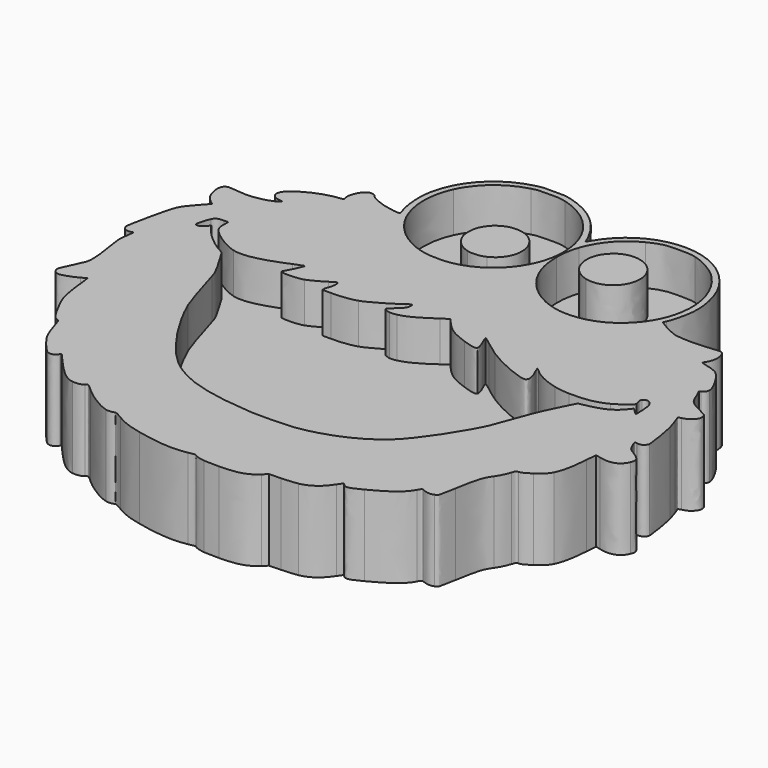
from build123d import *

# Parameters (mm, degrees)
F1_DEPTH = 30
F2_DEPTH = 15


# Not quite as in the source:
# - ends of sketch curves that miss each other by under 0.0002 mm in the source are joined


with BuildPart() as f1:
    # F0 (on Top) → F1 (new body)
    with BuildSketch(Plane.XY):
        with BuildLine():
            Line((-93.029528, 29.788683), (-95.476175, 27.033423))
            add(Edge.make_bspline(
                [(-99.819891, 21.007661), (-99.221413, 22.582728), (-98.328893, 23.820866), (-95.476175, 27.033423)],
                knots=[0, 0, 0, 0, 1, 1, 1, 1], degree=3))
            add(Edge.make_bspline(
                [(-103.713193, 3.050118), (-103.970353, 4.141773), (-100.969921, 17.981028), (-99.819891, 21.007661)],
                knots=[0, 0, 0, 0, 1, 1, 1, 1], degree=3))
            add(Edge.make_bspline(
                [(-100.414026, 1.339518), (-101.819569, 0.805128), (-103.374235, 1.611213), (-103.713193, 3.050118)],
                knots=[0, 0, 0, 0, 1, 1, 1, 1], degree=3))
            add(Edge.make_bspline(
                [(-99.647491, 1.526403), (-99.689153, 1.568103), (-100.034093, 1.483953), (-100.414026, 1.339518)],
                knots=[0, 0, 0, 0, 1, 1, 1, 1], degree=3))
            add(Edge.make_bspline(
                [(-99.944067, -1.180309), (-99.739289, 0.266726), (-99.60583, 1.484748), (-99.647491, 1.526403)],
                knots=[0, 0, 0, 0, 1, 1, 1, 1], degree=3))
            add(Edge.make_bspline(
                [(-99.28666, -11.536467), (-100.310645, -5.310492), (-100.378123, -4.247494), (-99.944067, -1.180309)],
                knots=[0, 0, 0, 0, 1, 1, 1, 1], degree=3))
            add(Edge.make_bspline(
                [(-98.923766, -21.571272), (-98.317863, -19.791319), (-98.427469, -16.760479), (-99.28666, -11.536467)],
                knots=[0, 0, 0, 0, 1, 1, 1, 1], degree=3))
            add(Edge.make_bspline(
                [(-101.044885, -26.305017), (-100.102937, -24.361459), (-99.148433, -22.231272), (-98.923766, -21.571272)],
                knots=[0, 0, 0, 0, 1, 1, 1, 1], degree=3))
            add(Edge.make_bspline(
                [(-102.533664, -30.722022), (-102.740319, -29.906629), (-102.625927, -29.567247), (-101.044885, -26.305017)],
                knots=[0, 0, 0, 0, 1, 1, 1, 1], degree=3))
            add(Edge.make_bspline(
                [(-100.234238, -32.539272), (-101.32717, -32.539272), (-102.259921, -31.802112), (-102.533664, -30.722022)],
                knots=[0, 0, 0, 0, 1, 1, 1, 1], degree=3))
            add(Edge.make_bspline(
                [(-93.938045, -30.319534), (-95.837959, -31.410252), (-99.040383, -32.539272), (-100.234238, -32.539272)],
                knots=[0, 0, 0, 0, 1, 1, 1, 1], degree=3))
            add(Edge.make_bspline(
                [(-92.121158, -29.371272), (-92.211975, -29.371272), (-93.029574, -29.797992), (-93.938045, -30.319534)],
                knots=[0, 0, 0, 0, 1, 1, 1, 1], degree=3))
            add(Edge.make_bspline(
                [(-91.660652, -32.311272), (-91.823114, -30.694272), (-92.030342, -29.371272), (-92.121158, -29.371272)],
                knots=[0, 0, 0, 0, 1, 1, 1, 1], degree=3))
            add(Edge.make_bspline(
                [(-86.11969, -51.113817), (-89.93609, -44.436724), (-90.704304, -41.829889), (-91.660652, -32.311272)],
                knots=[0, 0, 0, 0, 1, 1, 1, 1], degree=3))
            add(Edge.make_bspline(
                [(-82.710365, -55.155972), (-83.822815, -54.791457), (-84.427328, -54.074734), (-86.11969, -51.113817)],
                knots=[0, 0, 0, 0, 1, 1, 1, 1], degree=3))
            add(Edge.make_bspline(
                [(-81.015003, -58.411272), (-81.891619, -55.540977), (-81.964918, -55.400239), (-82.710365, -55.155972)],
                knots=[0, 0, 0, 0, 1, 1, 1, 1], degree=3))
            add(Edge.make_bspline(
                [(-77.687252, -66.438934), (-78.970304, -64.520614), (-79.649686, -62.881707), (-81.015003, -58.411272)],
                knots=[0, 0, 0, 0, 1, 1, 1, 1], degree=3))
            add(Edge.make_bspline(
                [(-72.258989, -72.746644), (-73.15899, -72.156942), (-76.31802, -68.486104), (-77.687252, -66.438934)],
                knots=[0, 0, 0, 0, 1, 1, 1, 1], degree=3))
            add(Edge.make_bspline(
                [(-68.552403, -71.629707), (-69.09577, -73.051092), (-70.944228, -73.608109), (-72.258989, -72.746644)],
                knots=[0, 0, 0, 0, 1, 1, 1, 1], degree=3))
            add(Edge.make_bspline(
                [(-68.023097, -71.389707), (-68.28392, -71.099502), (-68.363516, -71.135592), (-68.552403, -71.629707)],
                knots=[0, 0, 0, 0, 1, 1, 1, 1], degree=3))
            add(Edge.make_bspline(
                [(-65.017563, -74.785422), (-66.501764, -73.105639), (-67.854255, -71.577567), (-68.023097, -71.389707)],
                knots=[0, 0, 0, 0, 1, 1, 1, 1], degree=3))
            add(Edge.make_bspline(
                [(-54.969721, -82.808914), (-57.326718, -82.529764), (-60.207383, -80.229469), (-65.017563, -74.785422)],
                knots=[0, 0, 0, 0, 1, 1, 1, 1], degree=3))
            add(Edge.make_bspline(
                [(-50.826133, -82.011349), (-51.668437, -82.720099), (-53.211615, -83.017137), (-54.969721, -82.808914)],
                knots=[0, 0, 0, 0, 1, 1, 1, 1], degree=3))
            add(Edge.make_bspline(
                [(-47.324831, -83.775162), (-50.234641, -81.175542), (-49.983306, -81.302157), (-50.826133, -82.011349)],
                knots=[0, 0, 0, 0, 1, 1, 1, 1], degree=3))
            add(Edge.make_bspline(
                [(-36.18981, -90.530569), (-38.866944, -89.892739), (-43.884712, -86.848557), (-47.324831, -83.775162)],
                knots=[0, 0, 0, 0, 1, 1, 1, 1], degree=3))
            add(Edge.make_bspline(
                [(-33.024309, -90.218817), (-34.101746, -90.664602), (-35.181074, -90.770899), (-36.18981, -90.530569)],
                knots=[0, 0, 0, 0, 1, 1, 1, 1], degree=3))
            add(Edge.make_bspline(
                [(-29.88518, -91.707297), (-31.739233, -90.583962), (-32.749281, -90.105027), (-33.024309, -90.218817)],
                knots=[0, 0, 0, 0, 1, 1, 1, 1], degree=3))
            add(Edge.make_bspline(
                [(-19.869808, -95.462854), (-24.390538, -94.461147), (-26.881866, -93.526954), (-29.88518, -91.707297)],
                knots=[0, 0, 0, 0, 1, 1, 1, 1], degree=3))
            add(Edge.make_bspline(
                [(-0.78596, -96.777154), (-5.539228, -97.745764), (-11.383431, -97.343269), (-19.869808, -95.462854)],
                knots=[0, 0, 0, 0, 1, 1, 1, 1], degree=3))
            add(Edge.make_bspline(
                [(2.15359, -96.634827), (1.776407, -96.298212), (1.49824, -96.311682), (-0.78596, -96.777154)],
                knots=[0, 0, 0, 0, 1, 1, 1, 1], degree=3))
            add(Edge.make_bspline(
                [(6.050185, -97.787959), (4.144345, -97.509439), (2.632172, -97.061937), (2.15359, -96.634827)],
                knots=[0, 0, 0, 0, 1, 1, 1, 1], degree=3))
            add(Edge.make_bspline(
                [(11.690185, -97.900512), (9.314185, -97.944687), (6.776185, -97.893762), (6.050185, -97.787959)],
                knots=[0, 0, 0, 0, 1, 1, 1, 1], degree=3))
            add(Edge.make_bspline(
                [(24.452897, -94.094802), (21.433247, -96.921042), (18.578192, -97.772389), (11.690185, -97.900512)],
                knots=[0, 0, 0, 0, 1, 1, 1, 1], degree=3))
            Line((24.452897, -94.094802), (26.037947, -92.611272))
            Line((26.037947, -92.611272), (30.38407, -92.461924))
            add(Edge.make_bspline(
                [(36.530185, -91.918414), (35.464187, -92.151844), (32.957942, -92.373477), (30.38407, -92.461924)],
                knots=[0, 0, 0, 0, 1, 1, 1, 1], degree=3))
            add(Edge.make_bspline(
                [(45.390227, -85.448254), (42.857867, -89.215857), (40.28212, -91.096827), (36.530185, -91.918414)],
                knots=[0, 0, 0, 0, 1, 1, 1, 1], degree=3))
            Line((45.390227, -85.448254), (46.655875, -83.565244))
            Line((46.655875, -83.565244), (47.32141, -84.202864))
            add(Edge.make_bspline(
                [(53.727362, -82.902364), (49.401947, -85.145374), (48.496952, -85.329102), (47.32141, -84.202864)],
                knots=[0, 0, 0, 0, 1, 1, 1, 1], degree=3))
            add(Edge.make_bspline(
                [(65.773232, -73.567969), (64.130245, -76.658089), (60.8155, -79.226704), (53.727362, -82.902364)],
                knots=[0, 0, 0, 0, 1, 1, 1, 1], degree=3))
            add(Edge.make_bspline(
                [(66.973232, -72.226857), (66.663407, -72.094752), (66.400015, -72.389112), (65.773232, -73.567969)],
                knots=[0, 0, 0, 0, 1, 1, 1, 1], degree=3))
            add(Edge.make_bspline(
                [(71.678575, -72.711589), (70.355995, -73.264204), (69.103622, -73.135182), (66.973232, -72.226857)],
                knots=[0, 0, 0, 0, 1, 1, 1, 1], degree=3))
            add(Edge.make_bspline(
                [(72.76273, -71.865207), (72.613585, -72.143892), (72.12571, -72.524764), (71.678575, -72.711589)],
                knots=[0, 0, 0, 0, 1, 1, 1, 1], degree=3))
            add(Edge.make_bspline(
                [(73.991372, -65.784889), (73.464767, -68.850379), (72.911875, -71.586522), (72.76273, -71.865207)],
                knots=[0, 0, 0, 0, 1, 1, 1, 1], degree=3))
            add(Edge.make_bspline(
                [(77.930185, -52.891272), (75.960002, -55.616232), (75.453227, -57.275157), (73.991372, -65.784889)],
                knots=[0, 0, 0, 0, 1, 1, 1, 1], degree=3))
            add(Edge.make_bspline(
                [(80.420605, -47.838732), (79.775477, -49.800514), (78.941425, -51.492627), (77.930185, -52.891272)],
                knots=[0, 0, 0, 0, 1, 1, 1, 1], degree=3))
            add(Edge.make_bspline(
                [(81.737972, -46.243504), (80.970122, -46.265254), (80.916805, -46.329837), (80.420605, -47.838732)],
                knots=[0, 0, 0, 0, 1, 1, 1, 1], degree=3))
            add(Edge.make_bspline(
                [(85.849487, -44.275377), (83.516972, -45.808962), (82.66402, -46.217254), (81.737972, -46.243504)],
                knots=[0, 0, 0, 0, 1, 1, 1, 1], degree=3))
            add(Edge.make_bspline(
                [(90.029335, -39.972582), (89.163287, -41.688207), (88.065197, -42.818599), (85.849487, -44.275377)],
                knots=[0, 0, 0, 0, 1, 1, 1, 1], degree=3))
            add(Edge.make_bspline(
                [(92.461855, -27.934639), (92.026615, -33.925677), (91.322275, -37.411287), (90.029335, -39.972582)],
                knots=[0, 0, 0, 0, 1, 1, 1, 1], degree=3))
            add(Edge.make_bspline(
                [(92.82055, -24.074494), (92.7718, -24.153424), (92.610362, -25.890484), (92.461855, -27.934639)],
                knots=[0, 0, 0, 0, 1, 1, 1, 1], degree=3))
            add(Edge.make_bspline(
                [(94.659715, -24.385639), (93.696955, -24.135582), (92.86933, -23.995572), (92.82055, -24.074494)],
                knots=[0, 0, 0, 0, 1, 1, 1, 1], degree=3))
            add(Edge.make_bspline(
                [(103.38247, -21.098892), (102.010405, -24.382699), (99.006437, -25.514599), (94.659715, -24.385639)],
                knots=[0, 0, 0, 0, 1, 1, 1, 1], degree=3))
            add(Edge.make_bspline(
                [(100.370185, -16.092327), (103.641257, -18.105724), (104.226602, -19.078594), (103.38247, -21.098892)],
                knots=[0, 0, 0, 0, 1, 1, 1, 1], degree=3))
            add(Edge.make_bspline(
                [(97.567832, -13.283974), (98.274662, -14.723599), (98.478745, -14.928117), (100.370185, -16.092327)],
                knots=[0, 0, 0, 0, 1, 1, 1, 1], degree=3))
            add(Edge.make_bspline(
                [(96.644327, -11.081284), (96.732962, -11.438779), (97.148537, -12.429987), (97.567832, -13.283974)],
                knots=[0, 0, 0, 0, 1, 1, 1, 1], degree=3))
            add(Edge.make_bspline(
                [(97.266332, -10.655907), (96.499682, -10.436037), (96.486572, -10.444999), (96.644327, -11.081284)],
                knots=[0, 0, 0, 0, 1, 1, 1, 1], degree=3))
            add(Edge.make_bspline(
                [(100.503212, -8.866249), (100.23946, -10.272154), (98.766977, -11.086287), (97.266332, -10.655907)],
                knots=[0, 0, 0, 0, 1, 1, 1, 1], degree=3))
            add(Edge.make_bspline(
                [(98.65528, 2.980158), (99.432767, -0.202264), (100.656662, -8.048254), (100.503212, -8.866249)],
                knots=[0, 0, 0, 0, 1, 1, 1, 1], degree=3))
            add(Edge.make_bspline(
                [(97.34947, 7.058508), (97.800085, 5.910701), (98.387695, 4.075451), (98.65528, 2.980158)],
                knots=[0, 0, 0, 0, 1, 1, 1, 1], degree=3))
            add(Edge.make_bspline(
                [(96.530185, 9.317823), (96.530185, 9.223001), (96.898862, 8.206308), (97.34947, 7.058508)],
                knots=[0, 0, 0, 0, 1, 1, 1, 1], degree=3))
            add(Edge.make_bspline(
                [(97.550185, 9.750701), (96.989185, 9.607436), (96.530185, 9.412646), (96.530185, 9.317823)],
                knots=[0, 0, 0, 0, 1, 1, 1, 1], degree=3))
            add(Edge.make_bspline(
                [(100.82533, 11.460341), (99.859495, 10.494506), (99.281635, 10.192856), (97.550185, 9.750701)],
                knots=[0, 0, 0, 0, 1, 1, 1, 1], degree=3))
            add(Edge.make_bspline(
                [(101.78698, 14.752136), (102.192137, 13.589898), (101.877355, 12.512366), (100.82533, 11.460341)],
                knots=[0, 0, 0, 0, 1, 1, 1, 1], degree=3))
            add(Edge.make_bspline(
                [(98.581682, 16.952516), (101.145332, 15.704306), (101.552485, 15.424803), (101.78698, 14.752136)],
                knots=[0, 0, 0, 0, 1, 1, 1, 1], degree=3))
            add(Edge.make_bspline(
                [(92.794517, 22.051631), (93.650117, 19.783953), (94.74169, 18.822161), (98.581682, 16.952516)],
                knots=[0, 0, 0, 0, 1, 1, 1, 1], degree=3))
            add(Edge.make_bspline(
                [(91.568732, 24.932418), (91.882435, 24.303386), (92.434037, 23.007033), (92.794517, 22.051631)],
                knots=[0, 0, 0, 0, 1, 1, 1, 1], degree=3))
            Line((91.568732, 24.932418), (90.998357, 26.076108))
            Line((90.998357, 26.076108), (91.544275, 26.284871))
            add(Edge.make_bspline(
                [(93.028277, 28.567203), (93.052052, 27.474363), (92.521622, 26.658626), (91.544275, 26.284871)],
                knots=[0, 0, 0, 0, 1, 1, 1, 1], degree=3))
            add(Edge.make_bspline(
                [(87.312385, 38.291277), (89.535025, 36.525406), (92.982797, 30.659951), (93.028277, 28.567203)],
                knots=[0, 0, 0, 0, 1, 1, 1, 1], degree=3))
            add(Edge.make_bspline(
                [(81.451877, 40.468209), (84.649735, 39.640106), (86.461937, 38.966952), (87.312385, 38.291277)],
                knots=[0, 0, 0, 0, 1, 1, 1, 1], degree=3))
            Line((81.451877, 40.468209), (80.413562, 40.737086))
            Line((80.413562, 40.737086), (80.83858, 41.382905))
            add(Edge.make_bspline(
                [(82.08985, 47.064551), (82.482467, 45.109567), (82.07575, 43.262831), (80.83858, 41.382905)],
                knots=[0, 0, 0, 0, 1, 1, 1, 1], degree=3))
            add(Edge.make_bspline(
                [(79.807472, 49.588723), (80.96866, 49.588723), (81.758312, 48.715415), (82.08985, 47.064551)],
                knots=[0, 0, 0, 0, 1, 1, 1, 1], degree=3))
            add(Edge.make_bspline(
                [(75.824162, 49.202723), (77.56549, 49.415023), (79.357982, 49.588723), (79.807472, 49.588723)],
                knots=[0, 0, 0, 0, 1, 1, 1, 1], degree=3))
            add(Edge.make_bspline(
                [(63.115195, 49.540377), (65.06536, 48.832577), (71.406332, 48.664109), (75.824162, 49.202723)],
                knots=[0, 0, 0, 0, 1, 1, 1, 1], degree=3))
            add(Edge.make_bspline(
                [(57.235112, 52.444696), (58.943575, 51.339453), (61.11955, 50.264685), (63.115195, 49.540377)],
                knots=[0, 0, 0, 0, 1, 1, 1, 1], degree=3))
            Line((57.235112, 52.444696), (55.740032, 53.411891))
            Line((55.740032, 53.411891), (56.232947, 54.560308))
            add(Edge.make_bspline(
                [(58.607357, 66.028722), (58.607357, 62.768478), (57.536949, 57.598391), (56.232947, 54.560308)],
                knots=[0, 0, 0, 0, 1, 1, 1, 1], degree=3))
            add(Edge.make_bspline(
                [(55.626399, 78.748721), (57.404769, 75.034122), (58.607357, 69.902574), (58.607357, 66.028722)],
                knots=[0, 0, 0, 0, 1, 1, 1, 1], degree=3))
            add(Edge.make_bspline(
                [(43.490184, 91.32132), (48.617214, 88.679156), (53.091069, 84.044435), (55.626399, 78.748721)],
                knots=[0, 0, 0, 0, 1, 1, 1, 1], degree=3))
            add(Edge.make_bspline(
                [(7.442244, 80.380729), (14.629149, 93.11522), (30.602147, 97.963044), (43.490184, 91.32132)],
                knots=[0, 0, 0, 0, 1, 1, 1, 1], degree=3))
            add(Edge.make_bspline(
                [(6.290184, 79.373357), (6.290184, 78.768953), (6.768804, 79.187461), (7.442244, 80.380729)],
                knots=[0, 0, 0, 0, 1, 1, 1, 1], degree=3))
            add(Edge.make_bspline(
                [(2.965382, 85.757698), (4.302609, 83.80584), (6.290184, 79.989265), (6.290184, 79.373357)],
                knots=[0, 0, 0, 0, 1, 1, 1, 1], degree=3))
            add(Edge.make_bspline(
                [(-13.335321, 97.170458), (-6.666763, 95.402956), (-0.85484, 91.333799), (2.965382, 85.757698)],
                knots=[0, 0, 0, 0, 1, 1, 1, 1], degree=3))
            add(Edge.make_bspline(
                [(-20.349808, 97.91644), (-16.414296, 97.91644), (-15.972576, 97.86946), (-13.335321, 97.170458)],
                knots=[0, 0, 0, 0, 1, 1, 1, 1], degree=3))
            add(Edge.make_bspline(
                [(-27.412626, 97.158254), (-24.720538, 97.871225), (-24.299346, 97.91644), (-20.349808, 97.91644)],
                knots=[0, 0, 0, 0, 1, 1, 1, 1], degree=3))
            add(Edge.make_bspline(
                [(-43.580051, 85.877183), (-39.810222, 91.39487), (-34.08173, 95.392013), (-27.412626, 97.158254)],
                knots=[0, 0, 0, 0, 1, 1, 1, 1], degree=3))
            add(Edge.make_bspline(
                [(-48.096474, 75.268721), (-47.190632, 79.443517), (-45.892585, 82.492457), (-43.580051, 85.877183)],
                knots=[0, 0, 0, 0, 1, 1, 1, 1], degree=3))
            add(Edge.make_bspline(
                [(-47.12151, 60.658547), (-48.584425, 64.79176), (-49.004353, 71.084531), (-48.096474, 75.268721)],
                knots=[0, 0, 0, 0, 1, 1, 1, 1], degree=3))
            add(Edge.make_bspline(
                [(-46.74981, 59.363332), (-46.74981, 59.498104), (-46.917076, 60.080951), (-47.12151, 60.658547)],
                knots=[0, 0, 0, 0, 1, 1, 1, 1], degree=3))
            add(Edge.make_bspline(
                [(-52.591028, 60.024692), (-49.946243, 59.33752), (-46.74981, 58.97561), (-46.74981, 59.363332)],
                knots=[0, 0, 0, 0, 1, 1, 1, 1], degree=3))
            add(Edge.make_bspline(
                [(-59.19794, 63.036944), (-58.535463, 62.140898), (-55.620104, 60.811712), (-52.591028, 60.024692)],
                knots=[0, 0, 0, 0, 1, 1, 1, 1], degree=3))
            add(Edge.make_bspline(
                [(-62.209007, 63.686975), (-61.136941, 64.198208), (-59.851301, 63.920666), (-59.19794, 63.036944)],
                knots=[0, 0, 0, 0, 1, 1, 1, 1], degree=3))
            add(Edge.make_bspline(
                [(-65.211898, 57.33598), (-65.648638, 59.217114), (-63.921255, 62.870462), (-62.209007, 63.686975)],
                knots=[0, 0, 0, 0, 1, 1, 1, 1], degree=3))
            add(Edge.make_bspline(
                [(-66.489809, 55.724906), (-64.893029, 55.901421), (-64.882052, 55.915262), (-65.211898, 57.33598)],
                knots=[0, 0, 0, 0, 1, 1, 1, 1], degree=3))
            add(Edge.make_bspline(
                [(-80.419858, 49.936931), (-76.415038, 53.080178), (-71.340396, 55.188705), (-66.489809, 55.724906)],
                knots=[0, 0, 0, 0, 1, 1, 1, 1], degree=3))
            add(Edge.make_bspline(
                [(-81.790759, 44.909733), (-83.065027, 46.266129), (-82.511736, 48.295087), (-80.419858, 49.936931)],
                knots=[0, 0, 0, 0, 1, 1, 1, 1], degree=3))
            add(Edge.make_bspline(
                [(-78.836129, 43.828723), (-79.851029, 43.828723), (-81.259222, 44.343938), (-81.790759, 44.909733)],
                knots=[0, 0, 0, 0, 1, 1, 1, 1], degree=3))
            add(Edge.make_bspline(
                [(-79.673206, 42.508593), (-77.936979, 43.331179), (-77.621492, 43.828723), (-78.836129, 43.828723)],
                knots=[0, 0, 0, 0, 1, 1, 1, 1], degree=3))
            add(Edge.make_bspline(
                [(-92.361315, 40.723898), (-87.829944, 40.151061), (-83.306191, 40.787363), (-79.673206, 42.508593)],
                knots=[0, 0, 0, 0, 1, 1, 1, 1], degree=3))
            add(Edge.make_bspline(
                [(-95.6901, 41.009121), (-95.23894, 41.026664), (-93.740986, 40.898311), (-92.361315, 40.723898)],
                knots=[0, 0, 0, 0, 1, 1, 1, 1], degree=3))
            add(Edge.make_bspline(
                [(-97.514901, 35.923118), (-98.290613, 38.906539), (-97.562346, 40.936331), (-95.6901, 41.009121)],
                knots=[0, 0, 0, 0, 1, 1, 1, 1], degree=3))
            add(Edge.make_bspline(
                [(-93.829669, 30.385586), (-95.914982, 31.941228), (-96.841605, 33.333595), (-97.514901, 35.923118)],
                knots=[0, 0, 0, 0, 1, 1, 1, 1], degree=3))
            Line((-93.829669, 30.385586), (-93.029528, 29.788683))
        make_face()
        with BuildLine():
            Line((92.254809, 12.132933), (93.418967, 9.920831))
            add(Edge.make_bspline(
                [(96.523607, 2.217978), (96.144197, 3.910976), (94.71289, 7.462166), (93.418967, 9.920831)],
                knots=[0, 0, 0, 0, 1, 1, 1, 1], degree=3))
            add(Edge.make_bspline(
                [(98.208084, -7.972969), (98.205835, -7.345692), (96.90985, 0.494493), (96.523607, 2.217978)],
                knots=[0, 0, 0, 0, 1, 1, 1, 1], degree=3))
            add(Edge.make_bspline(
                [(96.350162, -7.537062), (98.175459, -8.516044), (98.210124, -8.524182), (98.208084, -7.972969)],
                knots=[0, 0, 0, 0, 1, 1, 1, 1], degree=3))
            add(Edge.make_bspline(
                [(93.338094, -5.325507), (94.005684, -6.028962), (95.272344, -6.958984), (96.350162, -7.537062)],
                knots=[0, 0, 0, 0, 1, 1, 1, 1], degree=3))
            add(Edge.make_bspline(
                [(93.317169, -8.294937), (92.012274, -3.689877), (92.010602, -3.926674), (93.338094, -5.325507)],
                knots=[0, 0, 0, 0, 1, 1, 1, 1], degree=3))
            add(Edge.make_bspline(
                [(97.785452, -17.268177), (96.188297, -16.466029), (94.898672, -13.876197), (93.317169, -8.294937)],
                knots=[0, 0, 0, 0, 1, 1, 1, 1], degree=3))
            add(Edge.make_bspline(
                [(101.327192, -19.771272), (101.325692, -19.427952), (99.46024, -18.109309), (97.785452, -17.268177)],
                knots=[0, 0, 0, 0, 1, 1, 1, 1], degree=3))
            add(Edge.make_bspline(
                [(99.720797, -22.010719), (100.422662, -21.652002), (101.329247, -20.388147), (101.327192, -19.771272)],
                knots=[0, 0, 0, 0, 1, 1, 1, 1], degree=3))
            add(Edge.make_bspline(
                [(92.50201, -21.153124), (96.203042, -22.647477), (98.046437, -22.866477), (99.720797, -22.010719)],
                knots=[0, 0, 0, 0, 1, 1, 1, 1], degree=3))
            add(Edge.make_bspline(
                [(90.65395, -20.527512), (90.701199, -20.480262), (91.532822, -20.761797), (92.50201, -21.153124)],
                knots=[0, 0, 0, 0, 1, 1, 1, 1], degree=3))
            add(Edge.make_bspline(
                [(90.1906, -26.555292), (90.398192, -23.287257), (90.606699, -20.574754), (90.65395, -20.527512)],
                knots=[0, 0, 0, 0, 1, 1, 1, 1], degree=3))
            add(Edge.make_bspline(
                [(85.398385, -41.707639), (88.640125, -39.421872), (89.557525, -36.521164), (90.1906, -26.555292)],
                knots=[0, 0, 0, 0, 1, 1, 1, 1], degree=3))
            add(Edge.make_bspline(
                [(81.569785, -43.850869), (81.759377, -44.040462), (83.36329, -43.142599), (85.398385, -41.707639)],
                knots=[0, 0, 0, 0, 1, 1, 1, 1], degree=3))
            add(Edge.make_bspline(
                [(81.410185, -41.931274), (81.410185, -42.899277), (81.482035, -43.763089), (81.569785, -43.850869)],
                knots=[0, 0, 0, 0, 1, 1, 1, 1], degree=3))
            add(Edge.make_bspline(
                [(81.209987, -40.171272), (81.320095, -40.171272), (81.410185, -40.963272), (81.410185, -41.931274)],
                knots=[0, 0, 0, 0, 1, 1, 1, 1], degree=3))
            add(Edge.make_bspline(
                [(78.398725, -46.411272), (79.143625, -44.090719), (80.909425, -40.171272), (81.209987, -40.171272)],
                knots=[0, 0, 0, 0, 1, 1, 1, 1], degree=3))
            add(Edge.make_bspline(
                [(75.516655, -52.280569), (77.224622, -49.660317), (77.603372, -48.889002), (78.398725, -46.411272)],
                knots=[0, 0, 0, 0, 1, 1, 1, 1], degree=3))
            add(Edge.make_bspline(
                [(72.671327, -60.019902), (73.485962, -55.935184), (73.94068, -54.698329), (75.516655, -52.280569)],
                knots=[0, 0, 0, 0, 1, 1, 1, 1], degree=3))
            add(Edge.make_bspline(
                [(70.850702, -70.471272), (70.852202, -70.054174), (72.10654, -62.851864), (72.671327, -60.019902)],
                knots=[0, 0, 0, 0, 1, 1, 1, 1], degree=3))
            add(Edge.make_bspline(
                [(68.53402, -70.298982), (69.050035, -70.660414), (70.849772, -70.794259), (70.850702, -70.471272)],
                knots=[0, 0, 0, 0, 1, 1, 1, 1], degree=3))
            add(Edge.make_bspline(
                [(67.752595, -68.798982), (67.911745, -69.454932), (68.24656, -70.097637), (68.53402, -70.298982)],
                knots=[0, 0, 0, 0, 1, 1, 1, 1], degree=3))
            add(Edge.make_bspline(
                [(66.320312, -65.131272), (66.52933, -65.131272), (67.40971, -67.385704), (67.752595, -68.798982)],
                knots=[0, 0, 0, 0, 1, 1, 1, 1], degree=3))
            add(Edge.make_bspline(
                [(65.644892, -67.147842), (65.93161, -66.038727), (66.235547, -65.131272), (66.320312, -65.131272)],
                knots=[0, 0, 0, 0, 1, 1, 1, 1], degree=3))
            add(Edge.make_bspline(
                [(60.399685, -76.127142), (62.953585, -74.266294), (64.48036, -71.652604), (65.644892, -67.147842)],
                knots=[0, 0, 0, 0, 1, 1, 1, 1], degree=3))
            add(Edge.make_bspline(
                [(49.13515, -82.376239), (49.476617, -82.717699), (57.346225, -78.351964), (60.399685, -76.127142)],
                knots=[0, 0, 0, 0, 1, 1, 1, 1], degree=3))
            add(Edge.make_bspline(
                [(49.857685, -79.298772), (49.380107, -80.911197), (49.054967, -82.296057), (49.13515, -82.376239)],
                knots=[0, 0, 0, 0, 1, 1, 1, 1], degree=3))
            add(Edge.make_bspline(
                [(50.595122, -76.236207), (50.667122, -76.308207), (50.335262, -77.686347), (49.857685, -79.298772)],
                knots=[0, 0, 0, 0, 1, 1, 1, 1], degree=3))
            add(Edge.make_bspline(
                [(46.314242, -79.842124), (47.241362, -78.695524), (50.396642, -76.037734), (50.595122, -76.236207)],
                knots=[0, 0, 0, 0, 1, 1, 1, 1], degree=3))
            add(Edge.make_bspline(
                [(43.662602, -83.645397), (44.672215, -82.108632), (45.86545, -80.397154), (46.314242, -79.842124)],
                knots=[0, 0, 0, 0, 1, 1, 1, 1], degree=3))
            add(Edge.make_bspline(
                [(40.798562, -87.335307), (41.364175, -86.842624), (42.65299, -85.182169), (43.662602, -83.645397)],
                knots=[0, 0, 0, 0, 1, 1, 1, 1], degree=3))
            add(Edge.make_bspline(
                [(30.050185, -90.088624), (35.631812, -90.066049), (38.510087, -89.328709), (40.798562, -87.335307)],
                knots=[0, 0, 0, 0, 1, 1, 1, 1], degree=3))
            add(Edge.make_bspline(
                [(25.664897, -90.312919), (26.162807, -90.197307), (28.136185, -90.096379), (30.050185, -90.088624)],
                knots=[0, 0, 0, 0, 1, 1, 1, 1], degree=3))
            add(Edge.make_bspline(
                [(23.11294, -92.076499), (24.236005, -91.017057), (25.047474, -90.456274), (25.664897, -90.312919)],
                knots=[0, 0, 0, 0, 1, 1, 1, 1], degree=3))
            add(Edge.make_bspline(
                [(17.450185, -95.132539), (19.613612, -94.702804), (21.285204, -93.800689), (23.11294, -92.076499)],
                knots=[0, 0, 0, 0, 1, 1, 1, 1], degree=3))
            add(Edge.make_bspline(
                [(5.750642, -95.365812), (7.582502, -95.654187), (15.632072, -95.493687), (17.450185, -95.132539)],
                knots=[0, 0, 0, 0, 1, 1, 1, 1], degree=3))
            add(Edge.make_bspline(
                [(3.411085, -94.342827), (3.409584, -94.775622), (4.201982, -95.122024), (5.750642, -95.365812)],
                knots=[0, 0, 0, 0, 1, 1, 1, 1], degree=3))
            add(Edge.make_bspline(
                [(3.88756, -93.271272), (3.62599, -93.700272), (3.41158, -94.182477), (3.411085, -94.342827)],
                knots=[0, 0, 0, 0, 1, 1, 1, 1], degree=3))
            add(Edge.make_bspline(
                [(4.23868, -92.491272), (4.307155, -92.491272), (4.149122, -92.842272), (3.88756, -93.271272)],
                knots=[0, 0, 0, 0, 1, 1, 1, 1], degree=3))
            add(Edge.make_bspline(
                [(2.936447, -93.088099), (3.58423, -92.759847), (4.170235, -92.491272), (4.23868, -92.491272)],
                knots=[0, 0, 0, 0, 1, 1, 1, 1], degree=3))
            add(Edge.make_bspline(
                [(-6.309808, -94.765932), (-1.61723, -94.771932), (0.30079, -94.423692), (2.936447, -93.088099)],
                knots=[0, 0, 0, 0, 1, 1, 1, 1], degree=3))
            add(Edge.make_bspline(
                [(-20.32574, -92.967522), (-15.067685, -94.251484), (-11.104603, -94.759999), (-6.309808, -94.765932)],
                knots=[0, 0, 0, 0, 1, 1, 1, 1], degree=3))
            add(Edge.make_bspline(
                [(-30.63401, -88.458147), (-26.24252, -91.196397), (-24.554128, -91.934982), (-20.32574, -92.967522)],
                knots=[0, 0, 0, 0, 1, 1, 1, 1], degree=3))
            add(Edge.make_bspline(
                [(-34.650129, -86.011272), (-34.599579, -86.011272), (-32.792322, -87.112369), (-30.63401, -88.458147)],
                knots=[0, 0, 0, 0, 1, 1, 1, 1], degree=3))
            add(Edge.make_bspline(
                [(-34.346973, -86.839744), (-34.564262, -86.384089), (-34.700682, -86.011272), (-34.650129, -86.011272)],
                knots=[0, 0, 0, 0, 1, 1, 1, 1], degree=3))
            add(Edge.make_bspline(
                [(-34.260244, -88.039744), (-34.006943, -87.734539), (-34.022423, -87.520332), (-34.346973, -86.839744)],
                knots=[0, 0, 0, 0, 1, 1, 1, 1], degree=3))
            add(Edge.make_bspline(
                [(-36.861942, -87.849477), (-35.242972, -88.507317), (-34.682325, -88.548319), (-34.260244, -88.039744)],
                knots=[0, 0, 0, 0, 1, 1, 1, 1], degree=3))
            add(Edge.make_bspline(
                [(-48.508508, -79.475674), (-43.064634, -84.320359), (-39.838286, -86.640079), (-36.861942, -87.849477)],
                knots=[0, 0, 0, 0, 1, 1, 1, 1], degree=3))
            add(Edge.make_bspline(
                [(-53.896453, -75.038794), (-53.8598, -74.874499), (-51.435224, -76.871097), (-48.508508, -79.475674)],
                knots=[0, 0, 0, 0, 1, 1, 1, 1], degree=3))
            add(Edge.make_bspline(
                [(-52.32482, -78.882147), (-52.969861, -78.205872), (-54.026531, -75.621844), (-53.896453, -75.038794)],
                knots=[0, 0, 0, 0, 1, 1, 1, 1], degree=3))
            Line((-52.32482, -78.882147), (-51.66981, -79.568869))
            Line((-51.66981, -79.568869), (-52.236397, -80.030067))
            add(Edge.make_bspline(
                [(-54.049409, -80.491272), (-53.176479, -80.491272), (-52.633206, -80.353077), (-52.236397, -80.030067)],
                knots=[0, 0, 0, 0, 1, 1, 1, 1], degree=3))
            add(Edge.make_bspline(
                [(-64.555755, -71.642247), (-58.363923, -78.745857), (-56.291615, -80.491272), (-54.049409, -80.491272)],
                knots=[0, 0, 0, 0, 1, 1, 1, 1], degree=3))
            add(Edge.make_bspline(
                [(-69.635784, -66.347284), (-69.507821, -65.926744), (-69.833861, -65.586912), (-64.555755, -71.642247)],
                knots=[0, 0, 0, 0, 1, 1, 1, 1], degree=3))
            add(Edge.make_bspline(
                [(-70.27848, -68.671272), (-69.982565, -67.582272), (-69.693353, -66.536479), (-69.635784, -66.347284)],
                knots=[0, 0, 0, 0, 1, 1, 1, 1], degree=3))
            add(Edge.make_bspline(
                [(-71.010557, -70.651272), (-70.903827, -70.651272), (-70.574393, -69.760272), (-70.27848, -68.671272)],
                knots=[0, 0, 0, 0, 1, 1, 1, 1], degree=3))
            add(Edge.make_bspline(
                [(-75.797652, -64.960197), (-74.599248, -66.779472), (-71.342453, -70.651272), (-71.010557, -70.651272)],
                knots=[0, 0, 0, 0, 1, 1, 1, 1], degree=3))
            add(Edge.make_bspline(
                [(-79.64586, -54.723702), (-77.89969, -60.894799), (-77.13407, -62.931402), (-75.797652, -64.960197)],
                knots=[0, 0, 0, 0, 1, 1, 1, 1], degree=3))
            Line((-79.64586, -54.723702), (-80.92698, -50.196132))
            Line((-80.92698, -50.196132), (-81.528031, -51.423702))
            add(Edge.make_bspline(
                [(-82.311595, -52.651272), (-82.211213, -52.651272), (-81.85861, -52.098867), (-81.528031, -51.423702)],
                knots=[0, 0, 0, 0, 1, 1, 1, 1], degree=3))
            add(Edge.make_bspline(
                [(-86.47232, -45.389517), (-85.034313, -48.391654), (-82.593706, -52.651272), (-82.311595, -52.651272)],
                knots=[0, 0, 0, 0, 1, 1, 1, 1], degree=3))
            add(Edge.make_bspline(
                [(-88.247901, -40.291272), (-87.899207, -42.023419), (-87.405112, -43.442119), (-86.47232, -45.389517)],
                knots=[0, 0, 0, 0, 1, 1, 1, 1], degree=3))
            add(Edge.make_bspline(
                [(-89.618969, -27.631272), (-89.393342, -32.175162), (-88.824654, -37.426242), (-88.247901, -40.291272)],
                knots=[0, 0, 0, 0, 1, 1, 1, 1], degree=3))
            add(Edge.make_bspline(
                [(-89.939239, -24.331272), (-89.853214, -24.331272), (-89.709092, -25.816272), (-89.618969, -27.631272)],
                knots=[0, 0, 0, 0, 1, 1, 1, 1], degree=3))
            add(Edge.make_bspline(
                [(-90.922728, -25.195422), (-90.467834, -24.720139), (-90.025264, -24.331272), (-89.939239, -24.331272)],
                knots=[0, 0, 0, 0, 1, 1, 1, 1], degree=3))
            add(Edge.make_bspline(
                [(-96.513728, -28.914942), (-94.16819, -27.789477), (-92.06869, -26.392744), (-90.922728, -25.195422)],
                knots=[0, 0, 0, 0, 1, 1, 1, 1], degree=3))
            add(Edge.make_bspline(
                [(-100.239587, -29.947909), (-100.433211, -30.391107), (-98.4364, -29.837509), (-96.513728, -28.914942)],
                knots=[0, 0, 0, 0, 1, 1, 1, 1], degree=3))
            add(Edge.make_bspline(
                [(-98.917869, -27.331279), (-99.592762, -28.651279), (-100.187535, -29.828757), (-100.239587, -29.947909)],
                knots=[0, 0, 0, 0, 1, 1, 1, 1], degree=3))
            add(Edge.make_bspline(
                [(-96.933902, -11.851279), (-95.664356, -19.340614), (-95.942672, -21.512187), (-98.917869, -27.331279)],
                knots=[0, 0, 0, 0, 1, 1, 1, 1], degree=3))
            add(Edge.make_bspline(
                [(-97.077122, 2.890878), (-97.947872, -3.585169), (-97.92433, -6.008517), (-96.933902, -11.851279)],
                knots=[0, 0, 0, 0, 1, 1, 1, 1], degree=3))
            add(Edge.make_bspline(
                [(-96.5409, 7.779813), (-96.482175, 7.721088), (-96.723474, 5.521068), (-97.077122, 2.890878)],
                knots=[0, 0, 0, 0, 1, 1, 1, 1], degree=3))
            add(Edge.make_bspline(
                [(-99.969808, 5.244573), (-97.914983, 6.961758), (-96.65468, 7.893596), (-96.5409, 7.779813)],
                knots=[0, 0, 0, 0, 1, 1, 1, 1], degree=3))
            add(Edge.make_bspline(
                [(-101.228064, 4.630166), (-101.229429, 4.284011), (-100.964322, 4.413468), (-99.969808, 5.244573)],
                knots=[0, 0, 0, 0, 1, 1, 1, 1], degree=3))
            add(Edge.make_bspline(
                [(-98.698578, 16.667186), (-99.544136, 13.439306), (-101.224839, 5.441373), (-101.228064, 4.630166)],
                knots=[0, 0, 0, 0, 1, 1, 1, 1], degree=3))
            add(Edge.make_bspline(
                [(-91.88069, 27.487826), (-97.273082, 21.690213), (-97.460828, 21.392246), (-98.698578, 16.667186)],
                knots=[0, 0, 0, 0, 1, 1, 1, 1], degree=3))
            add(Edge.make_bspline(
                [(-89.381434, 30.558371), (-89.23204, 30.508046), (-90.356705, 29.126336), (-91.88069, 27.487826)],
                knots=[0, 0, 0, 0, 1, 1, 1, 1], degree=3))
            add(Edge.make_bspline(
                [(-93.253307, 32.941604), (-92.407842, 32.297516), (-89.824911, 30.707658), (-89.381434, 30.558371)],
                knots=[0, 0, 0, 0, 1, 1, 1, 1], degree=3))
            add(Edge.make_bspline(
                [(-95.41302, 37.427238), (-95.255088, 35.685539), (-94.328234, 33.760502), (-93.253307, 32.941604)],
                knots=[0, 0, 0, 0, 1, 1, 1, 1], degree=3))
            Line((-95.41302, 37.427238), (-95.542556, 38.85579))
            Line((-95.542556, 38.85579), (-94.606182, 38.669478))
            add(Edge.make_bspline(
                [(-82.509809, 39.014684), (-85.766915, 38.190196), (-91.39076, 38.029703), (-94.606182, 38.669478)],
                knots=[0, 0, 0, 0, 1, 1, 1, 1], degree=3))
            add(Edge.make_bspline(
                [(-72.429809, 44.679721), (-72.429809, 43.555804), (-78.871028, 39.935788), (-82.509809, 39.014684)],
                knots=[0, 0, 0, 0, 1, 1, 1, 1], degree=3))
            add(Edge.make_bspline(
                [(-78.025774, 46.113428), (-74.16884, 45.786034), (-72.429809, 45.340489), (-72.429809, 44.679721)],
                knots=[0, 0, 0, 0, 1, 1, 1, 1], degree=3))
            add(Edge.make_bspline(
                [(-80.036136, 46.622905), (-79.942186, 46.378074), (-79.337158, 46.224743), (-78.025774, 46.113428)],
                knots=[0, 0, 0, 0, 1, 1, 1, 1], degree=3))
            add(Edge.make_bspline(
                [(-70.575687, 52.629241), (-75.153872, 51.056281), (-80.447659, 47.695314), (-80.036136, 46.622905)],
                knots=[0, 0, 0, 0, 1, 1, 1, 1], degree=3))
            add(Edge.make_bspline(
                [(-64.869809, 53.368532), (-68.251827, 53.282027), (-68.932347, 53.193855), (-70.575687, 52.629241)],
                knots=[0, 0, 0, 0, 1, 1, 1, 1], degree=3))
            add(Edge.make_bspline(
                [(-59.303465, 53.252749), (-60.252953, 53.370452), (-62.757809, 53.422553), (-64.869809, 53.368532)],
                knots=[0, 0, 0, 0, 1, 1, 1, 1], degree=3))
            add(Edge.make_bspline(
                [(-57.696785, 53.232371), (-57.630973, 53.125879), (-58.353975, 53.135049), (-59.303465, 53.252749)],
                knots=[0, 0, 0, 0, 1, 1, 1, 1], degree=3))
            add(Edge.make_bspline(
                [(-60.209063, 55.134222), (-58.893128, 54.194699), (-57.762603, 53.338867), (-57.696785, 53.232371)],
                knots=[0, 0, 0, 0, 1, 1, 1, 1], degree=3))
            add(Edge.make_bspline(
                [(-62.488532, 59.871776), (-63.553637, 57.769888), (-63.372037, 57.392454), (-60.209063, 55.134222)],
                knots=[0, 0, 0, 0, 1, 1, 1, 1], degree=3))
            add(Edge.make_bspline(
                [(-60.305785, 60.897383), (-61.315261, 61.783715), (-61.583562, 61.657648), (-62.488532, 59.871776)],
                knots=[0, 0, 0, 0, 1, 1, 1, 1], degree=3))
            add(Edge.make_bspline(
                [(-58.563137, 59.703184), (-59.054465, 59.949851), (-59.838659, 60.48724), (-60.305785, 60.897383)],
                knots=[0, 0, 0, 0, 1, 1, 1, 1], degree=3))
            add(Edge.make_bspline(
                [(-47.688412, 56.87231), (-50.776311, 57.096976), (-56.167137, 58.500302), (-58.563137, 59.703184)],
                knots=[0, 0, 0, 0, 1, 1, 1, 1], degree=3))
            Line((-47.688412, 56.87231), (-45.627016, 56.722326))
            Line((-45.627016, 56.722326), (-43.972612, 54.216815))
            add(Edge.make_bspline(
                [(-28.516993, 42.723487), (-34.70992, 44.520386), (-40.329224, 48.699083), (-43.972612, 54.216815)],
                knots=[0, 0, 0, 0, 1, 1, 1, 1], degree=3))
            add(Edge.make_bspline(
                [(-12.062675, 42.754979), (-17.973643, 41.049041), (-22.714775, 41.039969), (-28.516993, 42.723487)],
                knots=[0, 0, 0, 0, 1, 1, 1, 1], degree=3))
            add(Edge.make_bspline(
                [(3.431837, 54.44548), (-0.229828, 48.858461), (-6.00044, 44.50457), (-12.062675, 42.754979)],
                knots=[0, 0, 0, 0, 1, 1, 1, 1], degree=3))
            add(Edge.make_bspline(
                [(5.06956, 56.735392), (4.970207, 56.698724), (4.233235, 55.668263), (3.431837, 54.44548)],
                knots=[0, 0, 0, 0, 1, 1, 1, 1], degree=3))
            add(Edge.make_bspline(
                [(5.5576, 55.775392), (5.388527, 56.340062), (5.168905, 56.772062), (5.06956, 56.735392)],
                knots=[0, 0, 0, 0, 1, 1, 1, 1], degree=3))
            add(Edge.make_bspline(
                [(8.584862, 49.929424), (7.260497, 51.876367), (5.991017, 54.327873), (5.5576, 55.775392)],
                knots=[0, 0, 0, 0, 1, 1, 1, 1], degree=3))
            add(Edge.make_bspline(
                [(24.928585, 38.490655), (18.064172, 40.235623), (12.556967, 44.090049), (8.584862, 49.929424)],
                knots=[0, 0, 0, 0, 1, 1, 1, 1], degree=3))
            add(Edge.make_bspline(
                [(31.250162, 37.965168), (27.655525, 37.953333), (26.744372, 38.029076), (24.928585, 38.490655)],
                knots=[0, 0, 0, 0, 1, 1, 1, 1], degree=3))
            add(Edge.make_bspline(
                [(37.805327, 38.613883), (35.695735, 38.045196), (35.012237, 37.977554), (31.250162, 37.965168)],
                knots=[0, 0, 0, 0, 1, 1, 1, 1], degree=3))
            add(Edge.make_bspline(
                [(42.047912, 40.064777), (41.00983, 39.615972), (39.100667, 38.963069), (37.805327, 38.613883)],
                knots=[0, 0, 0, 0, 1, 1, 1, 1], degree=3))
            add(Edge.make_bspline(
                [(53.203697, 49.228723), (50.661805, 45.577601), (46.064965, 41.801517), (42.047912, 40.064777)],
                knots=[0, 0, 0, 0, 1, 1, 1, 1], degree=3))
            add(Edge.make_bspline(
                [(54.54064, 51.105631), (54.448607, 50.997331), (53.84698, 50.152723), (53.203697, 49.228723)],
                knots=[0, 0, 0, 0, 1, 1, 1, 1], degree=3))
            add(Edge.make_bspline(
                [(56.104832, 50.408983), (55.336562, 50.900438), (54.63268, 51.213931), (54.54064, 51.105631)],
                knots=[0, 0, 0, 0, 1, 1, 1, 1], degree=3))
            add(Edge.make_bspline(
                [(63.407522, 47.120745), (61.27561, 47.710893), (58.05718, 49.160081), (56.104832, 50.408983)],
                knots=[0, 0, 0, 0, 1, 1, 1, 1], degree=3))
            add(Edge.make_bspline(
                [(69.770162, 46.634899), (65.863412, 46.623619), (64.951922, 46.693226), (63.407522, 47.120745)],
                knots=[0, 0, 0, 0, 1, 1, 1, 1], degree=3))
            add(Edge.make_bspline(
                [(76.955672, 47.038915), (75.27916, 46.789331), (72.681947, 46.643301), (69.770162, 46.634899)],
                knots=[0, 0, 0, 0, 1, 1, 1, 1], degree=3))
            add(Edge.make_bspline(
                [(79.966487, 45.764495), (79.960487, 47.473809), (79.938812, 47.483015), (76.955672, 47.038915)],
                knots=[0, 0, 0, 0, 1, 1, 1, 1], degree=3))
            add(Edge.make_bspline(
                [(77.475512, 40.950599), (79.334695, 43.123322), (79.971362, 44.353689), (79.966487, 45.764495)],
                knots=[0, 0, 0, 0, 1, 1, 1, 1], degree=3))
            Line((77.475512, 40.950599), (75.936865, 39.152477))
            Line((75.936865, 39.152477), (79.09351, 38.525325))
            add(Edge.make_bspline(
                [(88.105345, 33.870578), (86.162582, 36.869078), (85.370395, 37.278254), (79.09351, 38.525325)],
                knots=[0, 0, 0, 0, 1, 1, 1, 1], degree=3))
            add(Edge.make_bspline(
                [(90.697345, 28.555908), (90.919645, 28.778201), (89.44282, 31.806303), (88.105345, 33.870578)],
                knots=[0, 0, 0, 0, 1, 1, 1, 1], degree=3))
            add(Edge.make_bspline(
                [(88.67683, 28.655388), (89.69935, 28.511906), (90.608582, 28.467138), (90.697345, 28.555908)],
                knots=[0, 0, 0, 0, 1, 1, 1, 1], degree=3))
            add(Edge.make_bspline(
                [(86.776735, 28.872498), (86.799235, 28.896573), (87.65431, 28.798848), (88.67683, 28.655388)],
                knots=[0, 0, 0, 0, 1, 1, 1, 1], degree=3))
            add(Edge.make_bspline(
                [(88.276015, 26.068721), (87.428875, 27.586721), (86.754205, 28.848423), (86.776735, 28.872498)],
                knots=[0, 0, 0, 0, 1, 1, 1, 1], degree=3))
            add(Edge.make_bspline(
                [(90.5887, 21.268721), (90.163862, 22.390721), (89.123154, 24.550721), (88.276015, 26.068721)],
                knots=[0, 0, 0, 0, 1, 1, 1, 1], degree=3))
            add(Edge.make_bspline(
                [(96.755492, 15.345933), (92.930859, 17.201996), (91.67002, 18.412953), (90.5887, 21.268721)],
                knots=[0, 0, 0, 0, 1, 1, 1, 1], degree=3))
            add(Edge.make_bspline(
                [(99.642392, 13.666143), (99.637892, 13.821566), (98.339005, 14.577468), (96.755492, 15.345933)],
                knots=[0, 0, 0, 0, 1, 1, 1, 1], degree=3))
            add(Edge.make_bspline(
                [(99.035169, 12.899808), (99.373412, 13.165871), (99.646659, 13.510721), (99.642392, 13.666143)],
                knots=[0, 0, 0, 0, 1, 1, 1, 1], degree=3))
            add(Edge.make_bspline(
                [(94.468045, 11.987553), (96.846429, 11.831321), (97.959437, 12.053628), (99.035169, 12.899808)],
                knots=[0, 0, 0, 0, 1, 1, 1, 1], degree=3))
            Line((94.468045, 11.987553), (92.254809, 12.132933))
        make_face(mode=Mode.SUBTRACT)
        with BuildLine():
            add(Edge.make_bspline(
                [(-15.609898, 44.191601), (-6.116945, 45.992383), (1.554302, 52.802051), (4.45651, 62.004292)],
                knots=[0, 0, 0, 0, 1, 1, 1, 1], degree=3))
            add(Edge.make_bspline(
                [(-25.239696, 44.201654), (-22.967668, 43.750209), (-17.964261, 43.744987), (-15.609898, 44.191601)],
                knots=[0, 0, 0, 0, 1, 1, 1, 1], degree=3))
            add(Edge.make_bspline(
                [(-42.739576, 56.515574), (-38.98865, 50.203624), (-32.512701, 45.646773), (-25.239696, 44.201654)],
                knots=[0, 0, 0, 0, 1, 1, 1, 1], degree=3))
            add(Edge.make_bspline(
                [(-44.005986, 80.683239), (-47.578209, 72.951632), (-47.101581, 63.85583), (-42.739576, 56.515574)],
                knots=[0, 0, 0, 0, 1, 1, 1, 1], degree=3))
            add(Edge.make_bspline(
                [(-26.656378, 95.119587), (-34.335676, 93.069164), (-40.74887, 87.732843), (-44.005986, 80.683239)],
                knots=[0, 0, 0, 0, 1, 1, 1, 1], degree=3))
            add(Edge.make_bspline(
                [(-20.349808, 95.746135), (-23.85932, 95.746135), (-24.576756, 95.674862), (-26.656378, 95.119587)],
                knots=[0, 0, 0, 0, 1, 1, 1, 1], degree=3))
            add(Edge.make_bspline(
                [(-14.043246, 95.119587), (-16.122861, 95.674859), (-16.840303, 95.746135), (-20.349808, 95.746135)],
                knots=[0, 0, 0, 0, 1, 1, 1, 1], degree=3))
            add(Edge.make_bspline(
                [(-2.439666, 88.648884), (-5.686985, 91.733523), (-9.660583, 93.949386), (-14.043246, 95.119587)],
                knots=[0, 0, 0, 0, 1, 1, 1, 1], degree=3))
            add(Edge.make_bspline(
                [(5.61058, 69.897512), (5.61133, 77.148721), (2.818765, 83.653891), (-2.439666, 88.648884)],
                knots=[0, 0, 0, 0, 1, 1, 1, 1], degree=3))
            add(Edge.make_bspline(
                [(4.45651, 62.004292), (5.311217, 64.714391), (5.610167, 66.759049), (5.61058, 69.897512)],
                knots=[0, 0, 0, 0, 1, 1, 1, 1], degree=3))
        make_face(mode=Mode.SUBTRACT)
        with BuildLine():
            add(Edge.make_bspline(
                [(37.085252, 40.811306), (46.017797, 43.077233), (53.085722, 50.186565), (55.475079, 59.308866)],
                knots=[0, 0, 0, 0, 1, 1, 1, 1], degree=3))
            add(Edge.make_bspline(
                [(27.950109, 40.228022), (30.356987, 39.888465), (34.486809, 40.152158), (37.085252, 40.811306)],
                knots=[0, 0, 0, 0, 1, 1, 1, 1], degree=3))
            add(Edge.make_bspline(
                [(14.009162, 47.051405), (17.849822, 43.349683), (22.720307, 40.96583), (27.950109, 40.228022)],
                knots=[0, 0, 0, 0, 1, 1, 1, 1], degree=3))
            add(Edge.make_bspline(
                [(6.028337, 66.127338), (6.020837, 58.582823), (8.707495, 52.161273), (14.009162, 47.051405)],
                knots=[0, 0, 0, 0, 1, 1, 1, 1], degree=3))
            add(Edge.make_bspline(
                [(7.413947, 74.872623), (6.466802, 72.234843), (6.031652, 69.488368), (6.028337, 66.127338)],
                knots=[0, 0, 0, 0, 1, 1, 1, 1], degree=3))
            add(Edge.make_bspline(
                [(20.330185, 89.563481), (14.234124, 86.564137), (9.801857, 81.522893), (7.413947, 74.872623)],
                knots=[0, 0, 0, 0, 1, 1, 1, 1], degree=3))
            add(Edge.make_bspline(
                [(31.130185, 91.920733), (25.965685, 91.920733), (24.447917, 91.589459), (20.330185, 89.563481)],
                knots=[0, 0, 0, 0, 1, 1, 1, 1], degree=3))
            add(Edge.make_bspline(
                [(37.349365, 91.394527), (35.718805, 91.846306), (34.839167, 91.920733), (31.130185, 91.920733)],
                knots=[0, 0, 0, 0, 1, 1, 1, 1], degree=3))
            add(Edge.make_bspline(
                [(49.149302, 84.325203), (46.51264, 87.238241), (41.490062, 90.247258), (37.349365, 91.394527)],
                knots=[0, 0, 0, 0, 1, 1, 1, 1], degree=3))
            add(Edge.make_bspline(
                [(55.475079, 59.308866), (57.784645, 68.126516), (55.448305, 77.36594), (49.149302, 84.325203)],
                knots=[0, 0, 0, 0, 1, 1, 1, 1], degree=3))
        make_face(mode=Mode.SUBTRACT)
        with BuildLine():
            add(Edge.make_bspline(
                [(96.523607, 2.217978), (96.144197, 3.910976), (94.71289, 7.462166), (93.418967, 9.920831)],
                knots=[0, 0, 0, 0, 1, 1, 1, 1], degree=3))
            Line((93.418967, 9.920831), (92.254809, 12.132933))
            Line((92.254809, 12.132933), (94.468045, 11.987553))
            add(Edge.make_bspline(
                [(94.468045, 11.987553), (96.846429, 11.831321), (97.959437, 12.053628), (99.035169, 12.899808)],
                knots=[0, 0, 0, 0, 1, 1, 1, 1], degree=3))
            add(Edge.make_bspline(
                [(99.035169, 12.899808), (99.373412, 13.165871), (99.646659, 13.510721), (99.642392, 13.666143)],
                knots=[0, 0, 0, 0, 1, 1, 1, 1], degree=3))
            add(Edge.make_bspline(
                [(99.642392, 13.666143), (99.637892, 13.821566), (98.339005, 14.577468), (96.755492, 15.345933)],
                knots=[0, 0, 0, 0, 1, 1, 1, 1], degree=3))
            add(Edge.make_bspline(
                [(96.755492, 15.345933), (92.930859, 17.201996), (91.67002, 18.412953), (90.5887, 21.268721)],
                knots=[0, 0, 0, 0, 1, 1, 1, 1], degree=3))
            add(Edge.make_bspline(
                [(90.5887, 21.268721), (90.163862, 22.390721), (89.123154, 24.550721), (88.276015, 26.068721)],
                knots=[0, 0, 0, 0, 1, 1, 1, 1], degree=3))
            add(Edge.make_bspline(
                [(88.276015, 26.068721), (87.428875, 27.586721), (86.754205, 28.848423), (86.776735, 28.872498)],
                knots=[0, 0, 0, 0, 1, 1, 1, 1], degree=3))
            add(Edge.make_bspline(
                [(86.776735, 28.872498), (86.799235, 28.896573), (87.65431, 28.798848), (88.67683, 28.655388)],
                knots=[0, 0, 0, 0, 1, 1, 1, 1], degree=3))
            add(Edge.make_bspline(
                [(88.67683, 28.655388), (89.69935, 28.511906), (90.608582, 28.467138), (90.697345, 28.555908)],
                knots=[0, 0, 0, 0, 1, 1, 1, 1], degree=3))
            add(Edge.make_bspline(
                [(90.697345, 28.555908), (90.919645, 28.778201), (89.44282, 31.806303), (88.105345, 33.870578)],
                knots=[0, 0, 0, 0, 1, 1, 1, 1], degree=3))
            add(Edge.make_bspline(
                [(88.105345, 33.870578), (86.162582, 36.869078), (85.370395, 37.278254), (79.09351, 38.525325)],
                knots=[0, 0, 0, 0, 1, 1, 1, 1], degree=3))
            Line((79.09351, 38.525325), (75.936865, 39.152477))
            Line((75.936865, 39.152477), (77.475512, 40.950599))
            add(Edge.make_bspline(
                [(77.475512, 40.950599), (79.334695, 43.123322), (79.971362, 44.353689), (79.966487, 45.764495)],
                knots=[0, 0, 0, 0, 1, 1, 1, 1], degree=3))
            add(Edge.make_bspline(
                [(79.966487, 45.764495), (79.960487, 47.473809), (79.938812, 47.483015), (76.955672, 47.038915)],
                knots=[0, 0, 0, 0, 1, 1, 1, 1], degree=3))
            add(Edge.make_bspline(
                [(76.955672, 47.038915), (75.27916, 46.789331), (72.681947, 46.643301), (69.770162, 46.634899)],
                knots=[0, 0, 0, 0, 1, 1, 1, 1], degree=3))
            add(Edge.make_bspline(
                [(69.770162, 46.634899), (65.863412, 46.623619), (64.951922, 46.693226), (63.407522, 47.120745)],
                knots=[0, 0, 0, 0, 1, 1, 1, 1], degree=3))
            add(Edge.make_bspline(
                [(63.407522, 47.120745), (61.27561, 47.710893), (58.05718, 49.160081), (56.104832, 50.408983)],
                knots=[0, 0, 0, 0, 1, 1, 1, 1], degree=3))
            add(Edge.make_bspline(
                [(56.104832, 50.408983), (55.336562, 50.900438), (54.63268, 51.213931), (54.54064, 51.105631)],
                knots=[0, 0, 0, 0, 1, 1, 1, 1], degree=3))
            add(Edge.make_bspline(
                [(54.54064, 51.105631), (54.448607, 50.997331), (53.84698, 50.152723), (53.203697, 49.228723)],
                knots=[0, 0, 0, 0, 1, 1, 1, 1], degree=3))
            add(Edge.make_bspline(
                [(53.203697, 49.228723), (50.661805, 45.577601), (46.064965, 41.801517), (42.047912, 40.064777)],
                knots=[0, 0, 0, 0, 1, 1, 1, 1], degree=3))
            add(Edge.make_bspline(
                [(42.047912, 40.064777), (41.00983, 39.615972), (39.100667, 38.963069), (37.805327, 38.613883)],
                knots=[0, 0, 0, 0, 1, 1, 1, 1], degree=3))
            add(Edge.make_bspline(
                [(37.805327, 38.613883), (35.695735, 38.045196), (35.012237, 37.977554), (31.250162, 37.965168)],
                knots=[0, 0, 0, 0, 1, 1, 1, 1], degree=3))
            add(Edge.make_bspline(
                [(31.250162, 37.965168), (27.655525, 37.953333), (26.744372, 38.029076), (24.928585, 38.490655)],
                knots=[0, 0, 0, 0, 1, 1, 1, 1], degree=3))
            add(Edge.make_bspline(
                [(24.928585, 38.490655), (18.064172, 40.235623), (12.556967, 44.090049), (8.584862, 49.929424)],
                knots=[0, 0, 0, 0, 1, 1, 1, 1], degree=3))
            add(Edge.make_bspline(
                [(8.584862, 49.929424), (7.260497, 51.876367), (5.991017, 54.327873), (5.5576, 55.775392)],
                knots=[0, 0, 0, 0, 1, 1, 1, 1], degree=3))
            add(Edge.make_bspline(
                [(5.5576, 55.775392), (5.388527, 56.340062), (5.168905, 56.772062), (5.06956, 56.735392)],
                knots=[0, 0, 0, 0, 1, 1, 1, 1], degree=3))
            add(Edge.make_bspline(
                [(5.06956, 56.735392), (4.970207, 56.698724), (4.233235, 55.668263), (3.431837, 54.44548)],
                knots=[0, 0, 0, 0, 1, 1, 1, 1], degree=3))
            add(Edge.make_bspline(
                [(3.431837, 54.44548), (-0.229828, 48.858461), (-6.00044, 44.50457), (-12.062675, 42.754979)],
                knots=[0, 0, 0, 0, 1, 1, 1, 1], degree=3))
            add(Edge.make_bspline(
                [(-12.062675, 42.754979), (-17.973643, 41.049041), (-22.714775, 41.039969), (-28.516993, 42.723487)],
                knots=[0, 0, 0, 0, 1, 1, 1, 1], degree=3))
            add(Edge.make_bspline(
                [(-28.516993, 42.723487), (-34.70992, 44.520386), (-40.329224, 48.699083), (-43.972612, 54.216815)],
                knots=[0, 0, 0, 0, 1, 1, 1, 1], degree=3))
            Line((-43.972612, 54.216815), (-45.627016, 56.722326))
            Line((-45.627016, 56.722326), (-47.688412, 56.87231))
            add(Edge.make_bspline(
                [(-47.688412, 56.87231), (-50.776311, 57.096976), (-56.167137, 58.500302), (-58.563137, 59.703184)],
                knots=[0, 0, 0, 0, 1, 1, 1, 1], degree=3))
            add(Edge.make_bspline(
                [(-58.563137, 59.703184), (-59.054465, 59.949851), (-59.838659, 60.48724), (-60.305785, 60.897383)],
                knots=[0, 0, 0, 0, 1, 1, 1, 1], degree=3))
            add(Edge.make_bspline(
                [(-60.305785, 60.897383), (-61.315261, 61.783715), (-61.583562, 61.657648), (-62.488532, 59.871776)],
                knots=[0, 0, 0, 0, 1, 1, 1, 1], degree=3))
            add(Edge.make_bspline(
                [(-62.488532, 59.871776), (-63.553637, 57.769888), (-63.372037, 57.392454), (-60.209063, 55.134222)],
                knots=[0, 0, 0, 0, 1, 1, 1, 1], degree=3))
            add(Edge.make_bspline(
                [(-60.209063, 55.134222), (-58.893128, 54.194699), (-57.762603, 53.338867), (-57.696785, 53.232371)],
                knots=[0, 0, 0, 0, 1, 1, 1, 1], degree=3))
            add(Edge.make_bspline(
                [(-57.696785, 53.232371), (-57.630973, 53.125879), (-58.353975, 53.135049), (-59.303465, 53.252749)],
                knots=[0, 0, 0, 0, 1, 1, 1, 1], degree=3))
            add(Edge.make_bspline(
                [(-59.303465, 53.252749), (-60.252953, 53.370452), (-62.757809, 53.422553), (-64.869809, 53.368532)],
                knots=[0, 0, 0, 0, 1, 1, 1, 1], degree=3))
            add(Edge.make_bspline(
                [(-64.869809, 53.368532), (-68.251827, 53.282027), (-68.932347, 53.193855), (-70.575687, 52.629241)],
                knots=[0, 0, 0, 0, 1, 1, 1, 1], degree=3))
            add(Edge.make_bspline(
                [(-70.575687, 52.629241), (-75.153872, 51.056281), (-80.447659, 47.695314), (-80.036136, 46.622905)],
                knots=[0, 0, 0, 0, 1, 1, 1, 1], degree=3))
            add(Edge.make_bspline(
                [(-80.036136, 46.622905), (-79.942186, 46.378074), (-79.337158, 46.224743), (-78.025774, 46.113428)],
                knots=[0, 0, 0, 0, 1, 1, 1, 1], degree=3))
            add(Edge.make_bspline(
                [(-78.025774, 46.113428), (-74.16884, 45.786034), (-72.429809, 45.340489), (-72.429809, 44.679721)],
                knots=[0, 0, 0, 0, 1, 1, 1, 1], degree=3))
            add(Edge.make_bspline(
                [(-72.429809, 44.679721), (-72.429809, 43.555804), (-78.871028, 39.935788), (-82.509809, 39.014684)],
                knots=[0, 0, 0, 0, 1, 1, 1, 1], degree=3))
            add(Edge.make_bspline(
                [(-82.509809, 39.014684), (-85.766915, 38.190196), (-91.39076, 38.029703), (-94.606182, 38.669478)],
                knots=[0, 0, 0, 0, 1, 1, 1, 1], degree=3))
            Line((-94.606182, 38.669478), (-95.542556, 38.85579))
            Line((-95.542556, 38.85579), (-95.41302, 37.427238))
            add(Edge.make_bspline(
                [(-95.41302, 37.427238), (-95.255088, 35.685539), (-94.328234, 33.760502), (-93.253307, 32.941604)],
                knots=[0, 0, 0, 0, 1, 1, 1, 1], degree=3))
            add(Edge.make_bspline(
                [(-93.253307, 32.941604), (-92.407842, 32.297516), (-89.824911, 30.707658), (-89.381434, 30.558371)],
                knots=[0, 0, 0, 0, 1, 1, 1, 1], degree=3))
            add(Edge.make_bspline(
                [(-89.381434, 30.558371), (-89.23204, 30.508046), (-90.356705, 29.126336), (-91.88069, 27.487826)],
                knots=[0, 0, 0, 0, 1, 1, 1, 1], degree=3))
            add(Edge.make_bspline(
                [(-91.88069, 27.487826), (-97.273082, 21.690213), (-97.460828, 21.392246), (-98.698578, 16.667186)],
                knots=[0, 0, 0, 0, 1, 1, 1, 1], degree=3))
            add(Edge.make_bspline(
                [(-98.698578, 16.667186), (-99.544136, 13.439306), (-101.224839, 5.441373), (-101.228064, 4.630166)],
                knots=[0, 0, 0, 0, 1, 1, 1, 1], degree=3))
            add(Edge.make_bspline(
                [(-101.228064, 4.630166), (-101.229429, 4.284011), (-100.964322, 4.413468), (-99.969808, 5.244573)],
                knots=[0, 0, 0, 0, 1, 1, 1, 1], degree=3))
            add(Edge.make_bspline(
                [(-99.969808, 5.244573), (-97.914983, 6.961758), (-96.65468, 7.893596), (-96.5409, 7.779813)],
                knots=[0, 0, 0, 0, 1, 1, 1, 1], degree=3))
            add(Edge.make_bspline(
                [(-96.5409, 7.779813), (-96.482175, 7.721088), (-96.723474, 5.521068), (-97.077122, 2.890878)],
                knots=[0, 0, 0, 0, 1, 1, 1, 1], degree=3))
            add(Edge.make_bspline(
                [(-97.077122, 2.890878), (-97.947872, -3.585169), (-97.92433, -6.008517), (-96.933902, -11.851279)],
                knots=[0, 0, 0, 0, 1, 1, 1, 1], degree=3))
            add(Edge.make_bspline(
                [(-96.933902, -11.851279), (-95.664356, -19.340614), (-95.942672, -21.512187), (-98.917869, -27.331279)],
                knots=[0, 0, 0, 0, 1, 1, 1, 1], degree=3))
            add(Edge.make_bspline(
                [(-98.917869, -27.331279), (-99.592762, -28.651279), (-100.187535, -29.828757), (-100.239587, -29.947909)],
                knots=[0, 0, 0, 0, 1, 1, 1, 1], degree=3))
            add(Edge.make_bspline(
                [(-100.239587, -29.947909), (-100.433211, -30.391107), (-98.4364, -29.837509), (-96.513728, -28.914942)],
                knots=[0, 0, 0, 0, 1, 1, 1, 1], degree=3))
            add(Edge.make_bspline(
                [(-96.513728, -28.914942), (-94.16819, -27.789477), (-92.06869, -26.392744), (-90.922728, -25.195422)],
                knots=[0, 0, 0, 0, 1, 1, 1, 1], degree=3))
            add(Edge.make_bspline(
                [(-90.922728, -25.195422), (-90.467834, -24.720139), (-90.025264, -24.331272), (-89.939239, -24.331272)],
                knots=[0, 0, 0, 0, 1, 1, 1, 1], degree=3))
            add(Edge.make_bspline(
                [(-89.939239, -24.331272), (-89.853214, -24.331272), (-89.709092, -25.816272), (-89.618969, -27.631272)],
                knots=[0, 0, 0, 0, 1, 1, 1, 1], degree=3))
            add(Edge.make_bspline(
                [(-89.618969, -27.631272), (-89.393342, -32.175162), (-88.824654, -37.426242), (-88.247901, -40.291272)],
                knots=[0, 0, 0, 0, 1, 1, 1, 1], degree=3))
            add(Edge.make_bspline(
                [(-88.247901, -40.291272), (-87.899207, -42.023419), (-87.405112, -43.442119), (-86.47232, -45.389517)],
                knots=[0, 0, 0, 0, 1, 1, 1, 1], degree=3))
            add(Edge.make_bspline(
                [(-86.47232, -45.389517), (-85.034313, -48.391654), (-82.593706, -52.651272), (-82.311595, -52.651272)],
                knots=[0, 0, 0, 0, 1, 1, 1, 1], degree=3))
            add(Edge.make_bspline(
                [(-82.311595, -52.651272), (-82.211213, -52.651272), (-81.85861, -52.098867), (-81.528031, -51.423702)],
                knots=[0, 0, 0, 0, 1, 1, 1, 1], degree=3))
            Line((-81.528031, -51.423702), (-80.92698, -50.196132))
            Line((-80.92698, -50.196132), (-79.64586, -54.723702))
            add(Edge.make_bspline(
                [(-79.64586, -54.723702), (-77.89969, -60.894799), (-77.13407, -62.931402), (-75.797652, -64.960197)],
                knots=[0, 0, 0, 0, 1, 1, 1, 1], degree=3))
            add(Edge.make_bspline(
                [(-75.797652, -64.960197), (-74.599248, -66.779472), (-71.342453, -70.651272), (-71.010557, -70.651272)],
                knots=[0, 0, 0, 0, 1, 1, 1, 1], degree=3))
            add(Edge.make_bspline(
                [(-71.010557, -70.651272), (-70.903827, -70.651272), (-70.574393, -69.760272), (-70.27848, -68.671272)],
                knots=[0, 0, 0, 0, 1, 1, 1, 1], degree=3))
            add(Edge.make_bspline(
                [(-70.27848, -68.671272), (-69.982565, -67.582272), (-69.693353, -66.536479), (-69.635784, -66.347284)],
                knots=[0, 0, 0, 0, 1, 1, 1, 1], degree=3))
            add(Edge.make_bspline(
                [(-69.635784, -66.347284), (-69.507821, -65.926744), (-69.833861, -65.586912), (-64.555755, -71.642247)],
                knots=[0, 0, 0, 0, 1, 1, 1, 1], degree=3))
            add(Edge.make_bspline(
                [(-64.555755, -71.642247), (-58.363923, -78.745857), (-56.291615, -80.491272), (-54.049409, -80.491272)],
                knots=[0, 0, 0, 0, 1, 1, 1, 1], degree=3))
            add(Edge.make_bspline(
                [(-54.049409, -80.491272), (-53.176479, -80.491272), (-52.633206, -80.353077), (-52.236397, -80.030067)],
                knots=[0, 0, 0, 0, 1, 1, 1, 1], degree=3))
            Line((-52.236397, -80.030067), (-51.66981, -79.568869))
            Line((-51.66981, -79.568869), (-52.32482, -78.882147))
            add(Edge.make_bspline(
                [(-52.32482, -78.882147), (-52.969861, -78.205872), (-54.026531, -75.621844), (-53.896453, -75.038794)],
                knots=[0, 0, 0, 0, 1, 1, 1, 1], degree=3))
            add(Edge.make_bspline(
                [(-53.896453, -75.038794), (-53.8598, -74.874499), (-51.435224, -76.871097), (-48.508508, -79.475674)],
                knots=[0, 0, 0, 0, 1, 1, 1, 1], degree=3))
            add(Edge.make_bspline(
                [(-48.508508, -79.475674), (-43.064634, -84.320359), (-39.838286, -86.640079), (-36.861942, -87.849477)],
                knots=[0, 0, 0, 0, 1, 1, 1, 1], degree=3))
            add(Edge.make_bspline(
                [(-36.861942, -87.849477), (-35.242972, -88.507317), (-34.682325, -88.548319), (-34.260244, -88.039744)],
                knots=[0, 0, 0, 0, 1, 1, 1, 1], degree=3))
            add(Edge.make_bspline(
                [(-34.260244, -88.039744), (-34.006943, -87.734539), (-34.022423, -87.520332), (-34.346973, -86.839744)],
                knots=[0, 0, 0, 0, 1, 1, 1, 1], degree=3))
            add(Edge.make_bspline(
                [(-34.346973, -86.839744), (-34.564262, -86.384089), (-34.700682, -86.011272), (-34.650129, -86.011272)],
                knots=[0, 0, 0, 0, 1, 1, 1, 1], degree=3))
            add(Edge.make_bspline(
                [(-34.650129, -86.011272), (-34.599579, -86.011272), (-32.792322, -87.112369), (-30.63401, -88.458147)],
                knots=[0, 0, 0, 0, 1, 1, 1, 1], degree=3))
            add(Edge.make_bspline(
                [(-30.63401, -88.458147), (-26.24252, -91.196397), (-24.554128, -91.934982), (-20.32574, -92.967522)],
                knots=[0, 0, 0, 0, 1, 1, 1, 1], degree=3))
            add(Edge.make_bspline(
                [(-20.32574, -92.967522), (-15.067685, -94.251484), (-11.104603, -94.759999), (-6.309808, -94.765932)],
                knots=[0, 0, 0, 0, 1, 1, 1, 1], degree=3))
            add(Edge.make_bspline(
                [(-6.309808, -94.765932), (-1.61723, -94.771932), (0.30079, -94.423692), (2.936447, -93.088099)],
                knots=[0, 0, 0, 0, 1, 1, 1, 1], degree=3))
            add(Edge.make_bspline(
                [(2.936447, -93.088099), (3.58423, -92.759847), (4.170235, -92.491272), (4.23868, -92.491272)],
                knots=[0, 0, 0, 0, 1, 1, 1, 1], degree=3))
            add(Edge.make_bspline(
                [(4.23868, -92.491272), (4.307155, -92.491272), (4.149122, -92.842272), (3.88756, -93.271272)],
                knots=[0, 0, 0, 0, 1, 1, 1, 1], degree=3))
            add(Edge.make_bspline(
                [(3.88756, -93.271272), (3.62599, -93.700272), (3.41158, -94.182477), (3.411085, -94.342827)],
                knots=[0, 0, 0, 0, 1, 1, 1, 1], degree=3))
            add(Edge.make_bspline(
                [(3.411085, -94.342827), (3.409584, -94.775622), (4.201982, -95.122024), (5.750642, -95.365812)],
                knots=[0, 0, 0, 0, 1, 1, 1, 1], degree=3))
            add(Edge.make_bspline(
                [(5.750642, -95.365812), (7.582502, -95.654187), (15.632072, -95.493687), (17.450185, -95.132539)],
                knots=[0, 0, 0, 0, 1, 1, 1, 1], degree=3))
            add(Edge.make_bspline(
                [(17.450185, -95.132539), (19.613612, -94.702804), (21.285204, -93.800689), (23.11294, -92.076499)],
                knots=[0, 0, 0, 0, 1, 1, 1, 1], degree=3))
            add(Edge.make_bspline(
                [(23.11294, -92.076499), (24.236005, -91.017057), (25.047474, -90.456274), (25.664897, -90.312919)],
                knots=[0, 0, 0, 0, 1, 1, 1, 1], degree=3))
            add(Edge.make_bspline(
                [(25.664897, -90.312919), (26.162807, -90.197307), (28.136185, -90.096379), (30.050185, -90.088624)],
                knots=[0, 0, 0, 0, 1, 1, 1, 1], degree=3))
            add(Edge.make_bspline(
                [(30.050185, -90.088624), (35.631812, -90.066049), (38.510087, -89.328709), (40.798562, -87.335307)],
                knots=[0, 0, 0, 0, 1, 1, 1, 1], degree=3))
            add(Edge.make_bspline(
                [(40.798562, -87.335307), (41.364175, -86.842624), (42.65299, -85.182169), (43.662602, -83.645397)],
                knots=[0, 0, 0, 0, 1, 1, 1, 1], degree=3))
            add(Edge.make_bspline(
                [(43.662602, -83.645397), (44.672215, -82.108632), (45.86545, -80.397154), (46.314242, -79.842124)],
                knots=[0, 0, 0, 0, 1, 1, 1, 1], degree=3))
            add(Edge.make_bspline(
                [(46.314242, -79.842124), (47.241362, -78.695524), (50.396642, -76.037734), (50.595122, -76.236207)],
                knots=[0, 0, 0, 0, 1, 1, 1, 1], degree=3))
            add(Edge.make_bspline(
                [(50.595122, -76.236207), (50.667122, -76.308207), (50.335262, -77.686347), (49.857685, -79.298772)],
                knots=[0, 0, 0, 0, 1, 1, 1, 1], degree=3))
            add(Edge.make_bspline(
                [(49.857685, -79.298772), (49.380107, -80.911197), (49.054967, -82.296057), (49.13515, -82.376239)],
                knots=[0, 0, 0, 0, 1, 1, 1, 1], degree=3))
            add(Edge.make_bspline(
                [(49.13515, -82.376239), (49.476617, -82.717699), (57.346225, -78.351964), (60.399685, -76.127142)],
                knots=[0, 0, 0, 0, 1, 1, 1, 1], degree=3))
            add(Edge.make_bspline(
                [(60.399685, -76.127142), (62.953585, -74.266294), (64.48036, -71.652604), (65.644892, -67.147842)],
                knots=[0, 0, 0, 0, 1, 1, 1, 1], degree=3))
            add(Edge.make_bspline(
                [(65.644892, -67.147842), (65.93161, -66.038727), (66.235547, -65.131272), (66.320312, -65.131272)],
                knots=[0, 0, 0, 0, 1, 1, 1, 1], degree=3))
            add(Edge.make_bspline(
                [(66.320312, -65.131272), (66.52933, -65.131272), (67.40971, -67.385704), (67.752595, -68.798982)],
                knots=[0, 0, 0, 0, 1, 1, 1, 1], degree=3))
            add(Edge.make_bspline(
                [(67.752595, -68.798982), (67.911745, -69.454932), (68.24656, -70.097637), (68.53402, -70.298982)],
                knots=[0, 0, 0, 0, 1, 1, 1, 1], degree=3))
            add(Edge.make_bspline(
                [(68.53402, -70.298982), (69.050035, -70.660414), (70.849772, -70.794259), (70.850702, -70.471272)],
                knots=[0, 0, 0, 0, 1, 1, 1, 1], degree=3))
            add(Edge.make_bspline(
                [(70.850702, -70.471272), (70.852202, -70.054174), (72.10654, -62.851864), (72.671327, -60.019902)],
                knots=[0, 0, 0, 0, 1, 1, 1, 1], degree=3))
            add(Edge.make_bspline(
                [(72.671327, -60.019902), (73.485962, -55.935184), (73.94068, -54.698329), (75.516655, -52.280569)],
                knots=[0, 0, 0, 0, 1, 1, 1, 1], degree=3))
            add(Edge.make_bspline(
                [(75.516655, -52.280569), (77.224622, -49.660317), (77.603372, -48.889002), (78.398725, -46.411272)],
                knots=[0, 0, 0, 0, 1, 1, 1, 1], degree=3))
            add(Edge.make_bspline(
                [(78.398725, -46.411272), (79.143625, -44.090719), (80.909425, -40.171272), (81.209987, -40.171272)],
                knots=[0, 0, 0, 0, 1, 1, 1, 1], degree=3))
            add(Edge.make_bspline(
                [(81.209987, -40.171272), (81.320095, -40.171272), (81.410185, -40.963272), (81.410185, -41.931274)],
                knots=[0, 0, 0, 0, 1, 1, 1, 1], degree=3))
            add(Edge.make_bspline(
                [(81.410185, -41.931274), (81.410185, -42.899277), (81.482035, -43.763089), (81.569785, -43.850869)],
                knots=[0, 0, 0, 0, 1, 1, 1, 1], degree=3))
            add(Edge.make_bspline(
                [(81.569785, -43.850869), (81.759377, -44.040462), (83.36329, -43.142599), (85.398385, -41.707639)],
                knots=[0, 0, 0, 0, 1, 1, 1, 1], degree=3))
            add(Edge.make_bspline(
                [(85.398385, -41.707639), (88.640125, -39.421872), (89.557525, -36.521164), (90.1906, -26.555292)],
                knots=[0, 0, 0, 0, 1, 1, 1, 1], degree=3))
            add(Edge.make_bspline(
                [(90.1906, -26.555292), (90.398192, -23.287257), (90.606699, -20.574754), (90.65395, -20.527512)],
                knots=[0, 0, 0, 0, 1, 1, 1, 1], degree=3))
            add(Edge.make_bspline(
                [(90.65395, -20.527512), (90.701199, -20.480262), (91.532822, -20.761797), (92.50201, -21.153124)],
                knots=[0, 0, 0, 0, 1, 1, 1, 1], degree=3))
            add(Edge.make_bspline(
                [(92.50201, -21.153124), (96.203042, -22.647477), (98.046437, -22.866477), (99.720797, -22.010719)],
                knots=[0, 0, 0, 0, 1, 1, 1, 1], degree=3))
            add(Edge.make_bspline(
                [(99.720797, -22.010719), (100.422662, -21.652002), (101.329247, -20.388147), (101.327192, -19.771272)],
                knots=[0, 0, 0, 0, 1, 1, 1, 1], degree=3))
            add(Edge.make_bspline(
                [(101.327192, -19.771272), (101.325692, -19.427952), (99.46024, -18.109309), (97.785452, -17.268177)],
                knots=[0, 0, 0, 0, 1, 1, 1, 1], degree=3))
            add(Edge.make_bspline(
                [(97.785452, -17.268177), (96.188297, -16.466029), (94.898672, -13.876197), (93.317169, -8.294937)],
                knots=[0, 0, 0, 0, 1, 1, 1, 1], degree=3))
            add(Edge.make_bspline(
                [(93.317169, -8.294937), (92.012274, -3.689877), (92.010602, -3.926674), (93.338094, -5.325507)],
                knots=[0, 0, 0, 0, 1, 1, 1, 1], degree=3))
            add(Edge.make_bspline(
                [(93.338094, -5.325507), (94.005684, -6.028962), (95.272344, -6.958984), (96.350162, -7.537062)],
                knots=[0, 0, 0, 0, 1, 1, 1, 1], degree=3))
            add(Edge.make_bspline(
                [(96.350162, -7.537062), (98.175459, -8.516044), (98.210124, -8.524182), (98.208084, -7.972969)],
                knots=[0, 0, 0, 0, 1, 1, 1, 1], degree=3))
            add(Edge.make_bspline(
                [(98.208084, -7.972969), (98.205835, -7.345692), (96.90985, 0.494493), (96.523607, 2.217978)],
                knots=[0, 0, 0, 0, 1, 1, 1, 1], degree=3))
        make_face()
        with BuildLine():
            add(Edge.make_bspline(
                [(-72.663332, 8.190146), (-76.076007, 9.799863), (-81.196527, 14.107931), (-83.461584, 17.275083)],
                knots=[0, 0, 0, 0, 1, 1, 1, 1], degree=3))
            Line((-83.461584, 17.275083), (-84.758946, 19.089146))
            Line((-84.758946, 19.089146), (-85.173944, 18.406728))
            add(Edge.make_bspline(
                [(-85.173944, 18.406728), (-86.230922, 16.668671), (-88.525, 15.849168), (-88.708515, 17.144096)],
                knots=[0, 0, 0, 0, 1, 1, 1, 1], degree=3))
            add(Edge.make_bspline(
                [(-88.708515, 17.144096), (-88.798497, 17.779031), (-87.97546, 20.638998), (-87.272214, 22.135091)],
                knots=[0, 0, 0, 0, 1, 1, 1, 1], degree=3))
            add(Edge.make_bspline(
                [(-87.272214, 22.135091), (-86.693199, 23.36689), (-85.981621, 23.699193), (-83.812958, 23.750553)],
                knots=[0, 0, 0, 0, 1, 1, 1, 1], degree=3))
            Line((-83.812958, 23.750553), (-82.200907, 23.788728))
            Line((-82.200907, 23.788728), (-82.251735, 21.904638))
            add(Edge.make_bspline(
                [(-82.251735, 21.904638), (-82.295212, 20.292813), (-82.210995, 19.833378), (-81.668919, 18.725425)],
                knots=[0, 0, 0, 0, 1, 1, 1, 1], degree=3))
            add(Edge.make_bspline(
                [(-81.668919, 18.725425), (-80.482627, 16.300728), (-73.822997, 11.850588), (-69.87517, 10.844531)],
                knots=[0, 0, 0, 0, 1, 1, 1, 1], degree=3))
            add(Edge.make_bspline(
                [(-69.87517, 10.844531), (-65.806056, 9.807558), (-60.082117, 11.023143), (-51.117801, 14.828005)],
                knots=[0, 0, 0, 0, 1, 1, 1, 1], degree=3))
            add(Edge.make_bspline(
                [(-51.117801, 14.828005), (-49.230195, 15.629193), (-47.633175, 16.232095), (-47.568867, 16.167783)],
                knots=[0, 0, 0, 0, 1, 1, 1, 1], degree=3))
            add(Edge.make_bspline(
                [(-47.568867, 16.167783), (-47.394846, 15.993768), (-49.313142, 11.725106), (-50.166705, 10.386986)],
                knots=[0, 0, 0, 0, 1, 1, 1, 1], degree=3))
            add(Edge.make_bspline(
                [(-50.166705, 10.386986), (-50.718738, 9.521568), (-50.83119, 9.17791), (-50.607573, 9.039708)],
                knots=[0, 0, 0, 0, 1, 1, 1, 1], degree=3))
            add(Edge.make_bspline(
                [(-50.607573, 9.039708), (-49.632519, 8.43709), (-44.306865, 8.641788), (-42.270844, 9.360145)],
                knots=[0, 0, 0, 0, 1, 1, 1, 1], degree=3))
            add(Edge.make_bspline(
                [(-42.270844, 9.360145), (-40.730853, 9.903483), (-38.380487, 11.15212), (-35.987973, 12.697923)],
                knots=[0, 0, 0, 0, 1, 1, 1, 1], degree=3))
            add(Edge.make_bspline(
                [(-35.987973, 12.697923), (-34.193968, 13.857033), (-33.703286, 14.078696), (-33.531648, 13.807556)],
                knots=[0, 0, 0, 0, 1, 1, 1, 1], degree=3))
            add(Edge.make_bspline(
                [(-33.531648, 13.807556), (-33.147918, 13.201368), (-33.289392, 11.046153), (-33.784542, 9.95494)],
                knots=[0, 0, 0, 0, 1, 1, 1, 1], degree=3))
            add(Edge.make_bspline(
                [(-33.784542, 9.95494), (-34.045644, 9.379525), (-34.261644, 8.611728), (-34.264542, 8.248728)],
                knots=[0, 0, 0, 0, 1, 1, 1, 1], degree=3))
            Line((-34.264542, 8.248728), (-34.269792, 7.588728))
            Line((-34.269792, 7.588728), (-30.969793, 7.589478))
            add(Edge.make_bspline(
                [(-30.969793, 7.589478), (-27.393283, 7.590228), (-24.046086, 8.031678), (-21.709446, 8.809968)],
                knots=[0, 0, 0, 0, 1, 1, 1, 1], degree=3))
            add(Edge.make_bspline(
                [(-21.709446, 8.809968), (-19.090618, 9.682255), (-13.586571, 12.855026), (-9.659728, 15.75595)],
                knots=[0, 0, 0, 0, 1, 1, 1, 1], degree=3))
            add(Edge.make_bspline(
                [(-9.659728, 15.75595), (-8.933923, 16.29214), (-8.234263, 16.665438), (-8.104933, 16.58551)],
                knots=[0, 0, 0, 0, 1, 1, 1, 1], degree=3))
            add(Edge.make_bspline(
                [(-8.104933, 16.58551), (-7.747536, 16.364628), (-7.823856, 15.077868), (-8.247276, 14.18557)],
                knots=[0, 0, 0, 0, 1, 1, 1, 1], degree=3))
            add(Edge.make_bspline(
                [(-8.247276, 14.18557), (-8.454891, 13.748058), (-9.291891, 12.824748), (-10.107276, 12.133765)],
                knots=[0, 0, 0, 0, 1, 1, 1, 1], degree=3))
            add(Edge.make_bspline(
                [(-10.107276, 12.133765), (-11.755138, 10.737325), (-12.429793, 10.038513), (-12.429793, 9.728095)],
                knots=[0, 0, 0, 0, 1, 1, 1, 1], degree=3))
            add(Edge.make_bspline(
                [(-12.429793, 9.728095), (-12.429793, 9.430593), (-11.257543, 8.879395), (-10.229166, 8.69335)],
                knots=[0, 0, 0, 0, 1, 1, 1, 1], degree=3))
            add(Edge.make_bspline(
                [(-10.229166, 8.69335), (-9.720793, 8.601378), (-8.608393, 8.6881), (-7.597611, 8.899113)],
                knots=[0, 0, 0, 0, 1, 1, 1, 1], degree=3))
            add(Edge.make_bspline(
                [(-7.597611, 8.899113), (-4.757616, 9.491268), (-1.345266, 11.284068), (3.694944, 14.832048)],
                knots=[0, 0, 0, 0, 1, 1, 1, 1], degree=3))
            add(Edge.make_bspline(
                [(3.694944, 14.832048), (4.973552, 15.732108), (6.107552, 16.46596), (6.214944, 16.46284)],
                knots=[0, 0, 0, 0, 1, 1, 1, 1], degree=3))
            add(Edge.make_bspline(
                [(6.214944, 16.46284), (6.322337, 16.45984), (6.734199, 16.017528), (7.130199, 15.48019)],
                knots=[0, 0, 0, 0, 1, 1, 1, 1], degree=3))
            add(Edge.make_bspline(
                [(7.130199, 15.48019), (7.526199, 14.942853), (8.678417, 13.71067), (9.690669, 12.742016)],
                knots=[0, 0, 0, 0, 1, 1, 1, 1], degree=3))
            add(Edge.make_bspline(
                [(9.690669, 12.742016), (11.729679, 10.790823), (13.502349, 9.825971), (18.220134, 8.099471)],
                knots=[0, 0, 0, 0, 1, 1, 1, 1], degree=3))
            add(Edge.make_bspline(
                [(18.220134, 8.099471), (21.443792, 6.919758), (23.479142, 6.591963), (23.717867, 7.214065)],
                knots=[0, 0, 0, 0, 1, 1, 1, 1], degree=3))
            add(Edge.make_bspline(
                [(23.717867, 7.214065), (23.926134, 7.756803), (23.490092, 9.20986), (22.434722, 11.48998)],
                knots=[0, 0, 0, 0, 1, 1, 1, 1], degree=3))
            add(Edge.make_bspline(
                [(22.434722, 11.48998), (21.960849, 12.513791), (21.637877, 13.416191), (21.717009, 13.495323)],
                knots=[0, 0, 0, 0, 1, 1, 1, 1], degree=3))
            add(Edge.make_bspline(
                [(21.717009, 13.495323), (21.796142, 13.574455), (23.028482, 12.721106), (24.455544, 11.598993)],
                knots=[0, 0, 0, 0, 1, 1, 1, 1], degree=3))
            add(Edge.make_bspline(
                [(24.455544, 11.598993), (25.882607, 10.476888), (28.292199, 8.718453), (29.810199, 7.691366)],
                knots=[0, 0, 0, 0, 1, 1, 1, 1], degree=3))
            add(Edge.make_bspline(
                [(29.810199, 7.691366), (34.571679, 4.469711), (43.905047, 0.388518), (46.511237, 0.388518)],
                knots=[0, 0, 0, 0, 1, 1, 1, 1], degree=3))
            add(Edge.make_bspline(
                [(46.511237, 0.388518), (47.924799, 0.388518), (47.874624, 2.396021), (46.381427, 5.582418)],
                knots=[0, 0, 0, 0, 1, 1, 1, 1], degree=3))
            add(Edge.make_bspline(
                [(46.381427, 5.582418), (45.847254, 6.72232), (45.410199, 7.761768), (45.410199, 7.892305)],
                knots=[0, 0, 0, 0, 1, 1, 1, 1], degree=3))
            add(Edge.make_bspline(
                [(45.410199, 7.892305), (45.410199, 8.02285), (45.896679, 7.681233), (46.491257, 7.13317)],
                knots=[0, 0, 0, 0, 1, 1, 1, 1], degree=3))
            add(Edge.make_bspline(
                [(46.491257, 7.13317), (48.929439, 4.885735), (52.054824, 3.353441), (56.690199, 2.13289)],
                knots=[0, 0, 0, 0, 1, 1, 1, 1], degree=3))
            add(Edge.make_bspline(
                [(56.690199, 2.13289), (58.409139, 1.680273), (59.810852, 1.502493), (62.386389, 1.410423)],
                knots=[0, 0, 0, 0, 1, 1, 1, 1], degree=3))
            add(Edge.make_bspline(
                [(62.386389, 1.410423), (68.112189, 1.205725), (72.132392, 1.940688), (75.883067, 3.877833)],
                knots=[0, 0, 0, 0, 1, 1, 1, 1], degree=3))
            add(Edge.make_bspline(
                [(75.883067, 3.877833), (78.464372, 5.211026), (81.982944, 7.972083), (81.800147, 8.521015)],
                knots=[0, 0, 0, 0, 1, 1, 1, 1], degree=3))
            add(Edge.make_bspline(
                [(81.800147, 8.521015), (81.112164, 10.586988), (81.080529, 10.895913), (81.492512, 11.524691)],
                knots=[0, 0, 0, 0, 1, 1, 1, 1], degree=3))
            add(Edge.make_bspline(
                [(81.492512, 11.524691), (82.105937, 12.460886), (83.548254, 12.409121), (84.379644, 11.421071)],
                knots=[0, 0, 0, 0, 1, 1, 1, 1], degree=3))
            add(Edge.make_bspline(
                [(84.379644, 11.421071), (84.716304, 11.020968), (85.1113, 10.291968), (85.257414, 9.801071)],
                knots=[0, 0, 0, 0, 1, 1, 1, 1], degree=3))
            add(Edge.make_bspline(
                [(85.257414, 9.801071), (85.59268, 8.674668), (85.867307, 3.508518), (85.591922, 3.508518)],
                knots=[0, 0, 0, 0, 1, 1, 1, 1], degree=3))
            add(Edge.make_bspline(
                [(85.591922, 3.508518), (85.479039, 3.508518), (84.866417, 4.02097), (84.230529, 4.647296)],
                knots=[0, 0, 0, 0, 1, 1, 1, 1], degree=3))
            Line((84.230529, 4.647296), (83.074375, 5.786066))
            Line((83.074375, 5.786066), (82.438862, 4.947296))
            add(Edge.make_bspline(
                [(82.438862, 4.947296), (79.742469, 1.388478), (76.916597, -0.160249), (70.909442, -1.371439)],
                knots=[0, 0, 0, 0, 1, 1, 1, 1], degree=3))
            Line((70.909442, -1.371439), (68.330199, -1.891474))
            Line((68.330199, -1.891474), (66.962057, -4.531475))
            add(Edge.make_bspline(
                [(66.962057, -4.531475), (64.206962, -9.847767), (61.97275, -14.973852), (60.162767, -20.131475)],
                knots=[0, 0, 0, 0, 1, 1, 1, 1], degree=3))
            add(Edge.make_bspline(
                [(60.162767, -20.131475), (57.347507, -28.153707), (56.610917, -29.886057), (54.244007, -34.051475)],
                knots=[0, 0, 0, 0, 1, 1, 1, 1], degree=3))
            add(Edge.make_bspline(
                [(54.244007, -34.051475), (49.719572, -42.013827), (44.49982, -49.272792), (40.672795, -52.92461)],
                knots=[0, 0, 0, 0, 1, 1, 1, 1], degree=3))
            add(Edge.make_bspline(
                [(40.672795, -52.92461), (34.441757, -58.87037), (24.274967, -63.42353), (13.610199, -65.044512)],
                knots=[0, 0, 0, 0, 1, 1, 1, 1], degree=3))
            add(Edge.make_bspline(
                [(13.610199, -65.044512), (11.312222, -65.393795), (0.826097, -65.6762), (-1.989793, -65.46464)],
                knots=[0, 0, 0, 0, 1, 1, 1, 1], degree=3))
            Line((-1.989793, -65.46464), (-1.989808, -65.464437))
            add(Edge.make_bspline(
                [(-1.989808, -65.464437), (-20.799613, -64.051264), (-30.467233, -61.072182), (-38.402428, -54.243874)],
                knots=[0, 0, 0, 0, 1, 1, 1, 1], degree=3))
            add(Edge.make_bspline(
                [(-38.402428, -54.243874), (-45.17128, -48.419224), (-53.994073, -35.381772), (-58.81977, -24.07316)],
                knots=[0, 0, 0, 0, 1, 1, 1, 1], degree=3))
            add(Edge.make_bspline(
                [(-58.81977, -24.07316), (-59.757253, -21.876252), (-61.709711, -15.762402), (-64.63893, -5.851272)],
                knots=[0, 0, 0, 0, 1, 1, 1, 1], degree=3))
            add(Edge.make_bspline(
                [(-64.63893, -5.851272), (-65.555718, -2.749287), (-65.390859, -3.064557), (-71.437364, 7.149798)],
                knots=[0, 0, 0, 0, 1, 1, 1, 1], degree=3))
            add(Edge.make_bspline(
                [(-71.437364, 7.149798), (-71.646084, 7.502388), (-72.19777, 7.970546), (-72.663332, 8.190146)],
                knots=[0, 0, 0, 0, 1, 1, 1, 1], degree=3))
        make_face(mode=Mode.SUBTRACT)
    extrude(amount=F1_DEPTH)


with BuildPart() as f1b:
    # F0 (on Top) → F1, piece 2 (new body)
    with BuildSketch(Plane.XY):
        with BuildLine():
            add(Edge.make_bspline(
                [(-16.743995, 53.078006), (-19.510475, 53.853969), (-21.710758, 55.714221), (-23.028808, 58.39156)],
                knots=[0, 0, 0, 0, 1, 1, 1, 1], degree=3))
            add(Edge.make_bspline(
                [(-9.925918, 53.625955), (-11.862095, 52.719907), (-14.664373, 52.494695), (-16.743995, 53.078006)],
                knots=[0, 0, 0, 0, 1, 1, 1, 1], degree=3))
            add(Edge.make_bspline(
                [(-6.771943, 69.444911), (-2.159803, 64.342547), (-3.717193, 56.531368), (-9.925918, 53.625955)],
                knots=[0, 0, 0, 0, 1, 1, 1, 1], degree=3))
            add(Edge.make_bspline(
                [(-22.285993, 68.227403), (-18.767075, 73.49702), (-10.986658, 74.107611), (-6.771943, 69.444911)],
                knots=[0, 0, 0, 0, 1, 1, 1, 1], degree=3))
            add(Edge.make_bspline(
                [(-23.904928, 62.06187), (-24.028423, 64.644914), (-23.60729, 66.24874), (-22.285993, 68.227403)],
                knots=[0, 0, 0, 0, 1, 1, 1, 1], degree=3))
            add(Edge.make_bspline(
                [(-23.028808, 58.39156), (-23.678728, 59.711735), (-23.821078, 60.30807), (-23.904928, 62.06187)],
                knots=[0, 0, 0, 0, 1, 1, 1, 1], degree=3))
        make_face()
    extrude(amount=F1_DEPTH)


with BuildPart() as f1c:
    # F0 (on Top) → F1, piece 3 (new body)
    with BuildSketch(Plane.XY):
        with BuildLine():
            add(Edge.make_bspline(
                [(21.195302, 60.768527), (14.995405, 62.435774), (12.007187, 69.119826), (14.85844, 74.942843)],
                knots=[0, 0, 0, 0, 1, 1, 1, 1], degree=3))
            add(Edge.make_bspline(
                [(33.650185, 70.367003), (33.650185, 63.891054), (27.42472, 59.093342), (21.195302, 60.768527)],
                knots=[0, 0, 0, 0, 1, 1, 1, 1], degree=3))
            add(Edge.make_bspline(
                [(19.894097, 79.597347), (26.555319, 82.150745), (33.650185, 77.390081), (33.650185, 70.367003)],
                knots=[0, 0, 0, 0, 1, 1, 1, 1], degree=3))
            add(Edge.make_bspline(
                [(14.85844, 74.942843), (15.737987, 76.739105), (18.07651, 78.900623), (19.894097, 79.597347)],
                knots=[0, 0, 0, 0, 1, 1, 1, 1], degree=3))
        make_face()
    extrude(amount=F1_DEPTH)


with BuildPart() as f2:
    # F0 (on Top) → F2 (new body)
    with BuildSketch(Plane.XY):
        with BuildLine():
            Line((-84.758946, 19.089146), (-83.461584, 17.275083))
            add(Edge.make_bspline(
                [(-72.663332, 8.190146), (-76.076007, 9.799863), (-81.196527, 14.107931), (-83.461584, 17.275083)],
                knots=[0, 0, 0, 0, 1, 1, 1, 1], degree=3))
            add(Edge.make_bspline(
                [(-71.437364, 7.149798), (-71.646084, 7.502388), (-72.19777, 7.970546), (-72.663332, 8.190146)],
                knots=[0, 0, 0, 0, 1, 1, 1, 1], degree=3))
            add(Edge.make_bspline(
                [(-64.63893, -5.851272), (-65.555718, -2.749287), (-65.390859, -3.064557), (-71.437364, 7.149798)],
                knots=[0, 0, 0, 0, 1, 1, 1, 1], degree=3))
            add(Edge.make_bspline(
                [(-58.81977, -24.07316), (-59.757253, -21.876252), (-61.709711, -15.762402), (-64.63893, -5.851272)],
                knots=[0, 0, 0, 0, 1, 1, 1, 1], degree=3))
            add(Edge.make_bspline(
                [(-38.402428, -54.243874), (-45.17128, -48.419224), (-53.994073, -35.381772), (-58.81977, -24.07316)],
                knots=[0, 0, 0, 0, 1, 1, 1, 1], degree=3))
            add(Edge.make_bspline(
                [(-1.989808, -65.464437), (-20.799613, -64.051264), (-30.467233, -61.072182), (-38.402428, -54.243874)],
                knots=[0, 0, 0, 0, 1, 1, 1, 1], degree=3))
            Line((-1.989808, -65.464437), (-1.989793, -65.46464))
            add(Edge.make_bspline(
                [(13.610199, -65.044512), (11.312222, -65.393795), (0.826097, -65.6762), (-1.989793, -65.46464)],
                knots=[0, 0, 0, 0, 1, 1, 1, 1], degree=3))
            add(Edge.make_bspline(
                [(40.672795, -52.92461), (34.441757, -58.87037), (24.274967, -63.42353), (13.610199, -65.044512)],
                knots=[0, 0, 0, 0, 1, 1, 1, 1], degree=3))
            add(Edge.make_bspline(
                [(54.244007, -34.051475), (49.719572, -42.013827), (44.49982, -49.272792), (40.672795, -52.92461)],
                knots=[0, 0, 0, 0, 1, 1, 1, 1], degree=3))
            add(Edge.make_bspline(
                [(60.162767, -20.131475), (57.347507, -28.153707), (56.610917, -29.886057), (54.244007, -34.051475)],
                knots=[0, 0, 0, 0, 1, 1, 1, 1], degree=3))
            add(Edge.make_bspline(
                [(66.962057, -4.531475), (64.206962, -9.847767), (61.97275, -14.973852), (60.162767, -20.131475)],
                knots=[0, 0, 0, 0, 1, 1, 1, 1], degree=3))
            Line((66.962057, -4.531475), (68.330199, -1.891474))
            Line((68.330199, -1.891474), (70.909442, -1.371439))
            add(Edge.make_bspline(
                [(82.438862, 4.947296), (79.742469, 1.388478), (76.916597, -0.160249), (70.909442, -1.371439)],
                knots=[0, 0, 0, 0, 1, 1, 1, 1], degree=3))
            Line((82.438862, 4.947296), (83.074375, 5.786066))
            Line((83.074375, 5.786066), (84.230529, 4.647296))
            add(Edge.make_bspline(
                [(85.591922, 3.508518), (85.479039, 3.508518), (84.866417, 4.02097), (84.230529, 4.647296)],
                knots=[0, 0, 0, 0, 1, 1, 1, 1], degree=3))
            add(Edge.make_bspline(
                [(85.257414, 9.801071), (85.59268, 8.674668), (85.867307, 3.508518), (85.591922, 3.508518)],
                knots=[0, 0, 0, 0, 1, 1, 1, 1], degree=3))
            add(Edge.make_bspline(
                [(84.379644, 11.421071), (84.716304, 11.020968), (85.1113, 10.291968), (85.257414, 9.801071)],
                knots=[0, 0, 0, 0, 1, 1, 1, 1], degree=3))
            add(Edge.make_bspline(
                [(81.492512, 11.524691), (82.105937, 12.460886), (83.548254, 12.409121), (84.379644, 11.421071)],
                knots=[0, 0, 0, 0, 1, 1, 1, 1], degree=3))
            add(Edge.make_bspline(
                [(81.800147, 8.521015), (81.112164, 10.586988), (81.080529, 10.895913), (81.492512, 11.524691)],
                knots=[0, 0, 0, 0, 1, 1, 1, 1], degree=3))
            add(Edge.make_bspline(
                [(75.883067, 3.877833), (78.464372, 5.211026), (81.982944, 7.972083), (81.800147, 8.521015)],
                knots=[0, 0, 0, 0, 1, 1, 1, 1], degree=3))
            add(Edge.make_bspline(
                [(62.386389, 1.410423), (68.112189, 1.205725), (72.132392, 1.940688), (75.883067, 3.877833)],
                knots=[0, 0, 0, 0, 1, 1, 1, 1], degree=3))
            add(Edge.make_bspline(
                [(56.690199, 2.13289), (58.409139, 1.680273), (59.810852, 1.502493), (62.386389, 1.410423)],
                knots=[0, 0, 0, 0, 1, 1, 1, 1], degree=3))
            add(Edge.make_bspline(
                [(46.491257, 7.13317), (48.929439, 4.885735), (52.054824, 3.353441), (56.690199, 2.13289)],
                knots=[0, 0, 0, 0, 1, 1, 1, 1], degree=3))
            add(Edge.make_bspline(
                [(45.410199, 7.892305), (45.410199, 8.02285), (45.896679, 7.681233), (46.491257, 7.13317)],
                knots=[0, 0, 0, 0, 1, 1, 1, 1], degree=3))
            add(Edge.make_bspline(
                [(46.381427, 5.582418), (45.847254, 6.72232), (45.410199, 7.761768), (45.410199, 7.892305)],
                knots=[0, 0, 0, 0, 1, 1, 1, 1], degree=3))
            add(Edge.make_bspline(
                [(46.511237, 0.388518), (47.924799, 0.388518), (47.874624, 2.396021), (46.381427, 5.582418)],
                knots=[0, 0, 0, 0, 1, 1, 1, 1], degree=3))
            add(Edge.make_bspline(
                [(29.810199, 7.691366), (34.571679, 4.469711), (43.905047, 0.388518), (46.511237, 0.388518)],
                knots=[0, 0, 0, 0, 1, 1, 1, 1], degree=3))
            add(Edge.make_bspline(
                [(24.455544, 11.598993), (25.882607, 10.476888), (28.292199, 8.718453), (29.810199, 7.691366)],
                knots=[0, 0, 0, 0, 1, 1, 1, 1], degree=3))
            add(Edge.make_bspline(
                [(21.717009, 13.495323), (21.796142, 13.574455), (23.028482, 12.721106), (24.455544, 11.598993)],
                knots=[0, 0, 0, 0, 1, 1, 1, 1], degree=3))
            add(Edge.make_bspline(
                [(22.434722, 11.48998), (21.960849, 12.513791), (21.637877, 13.416191), (21.717009, 13.495323)],
                knots=[0, 0, 0, 0, 1, 1, 1, 1], degree=3))
            add(Edge.make_bspline(
                [(23.717867, 7.214065), (23.926134, 7.756803), (23.490092, 9.20986), (22.434722, 11.48998)],
                knots=[0, 0, 0, 0, 1, 1, 1, 1], degree=3))
            add(Edge.make_bspline(
                [(18.220134, 8.099471), (21.443792, 6.919758), (23.479142, 6.591963), (23.717867, 7.214065)],
                knots=[0, 0, 0, 0, 1, 1, 1, 1], degree=3))
            add(Edge.make_bspline(
                [(9.690669, 12.742016), (11.729679, 10.790823), (13.502349, 9.825971), (18.220134, 8.099471)],
                knots=[0, 0, 0, 0, 1, 1, 1, 1], degree=3))
            add(Edge.make_bspline(
                [(7.130199, 15.48019), (7.526199, 14.942853), (8.678417, 13.71067), (9.690669, 12.742016)],
                knots=[0, 0, 0, 0, 1, 1, 1, 1], degree=3))
            add(Edge.make_bspline(
                [(6.214944, 16.46284), (6.322337, 16.45984), (6.734199, 16.017528), (7.130199, 15.48019)],
                knots=[0, 0, 0, 0, 1, 1, 1, 1], degree=3))
            add(Edge.make_bspline(
                [(3.694944, 14.832048), (4.973552, 15.732108), (6.107552, 16.46596), (6.214944, 16.46284)],
                knots=[0, 0, 0, 0, 1, 1, 1, 1], degree=3))
            add(Edge.make_bspline(
                [(-7.597611, 8.899113), (-4.757616, 9.491268), (-1.345266, 11.284068), (3.694944, 14.832048)],
                knots=[0, 0, 0, 0, 1, 1, 1, 1], degree=3))
            add(Edge.make_bspline(
                [(-10.229166, 8.69335), (-9.720793, 8.601378), (-8.608393, 8.6881), (-7.597611, 8.899113)],
                knots=[0, 0, 0, 0, 1, 1, 1, 1], degree=3))
            add(Edge.make_bspline(
                [(-12.429793, 9.728095), (-12.429793, 9.430593), (-11.257543, 8.879395), (-10.229166, 8.69335)],
                knots=[0, 0, 0, 0, 1, 1, 1, 1], degree=3))
            add(Edge.make_bspline(
                [(-10.107276, 12.133765), (-11.755138, 10.737325), (-12.429793, 10.038513), (-12.429793, 9.728095)],
                knots=[0, 0, 0, 0, 1, 1, 1, 1], degree=3))
            add(Edge.make_bspline(
                [(-8.247276, 14.18557), (-8.454891, 13.748058), (-9.291891, 12.824748), (-10.107276, 12.133765)],
                knots=[0, 0, 0, 0, 1, 1, 1, 1], degree=3))
            add(Edge.make_bspline(
                [(-8.104933, 16.58551), (-7.747536, 16.364628), (-7.823856, 15.077868), (-8.247276, 14.18557)],
                knots=[0, 0, 0, 0, 1, 1, 1, 1], degree=3))
            add(Edge.make_bspline(
                [(-9.659728, 15.75595), (-8.933923, 16.29214), (-8.234263, 16.665438), (-8.104933, 16.58551)],
                knots=[0, 0, 0, 0, 1, 1, 1, 1], degree=3))
            add(Edge.make_bspline(
                [(-21.709446, 8.809968), (-19.090618, 9.682255), (-13.586571, 12.855026), (-9.659728, 15.75595)],
                knots=[0, 0, 0, 0, 1, 1, 1, 1], degree=3))
            add(Edge.make_bspline(
                [(-30.969793, 7.589478), (-27.393283, 7.590228), (-24.046086, 8.031678), (-21.709446, 8.809968)],
                knots=[0, 0, 0, 0, 1, 1, 1, 1], degree=3))
            Line((-30.969793, 7.589478), (-34.269792, 7.588728))
            Line((-34.269792, 7.588728), (-34.264542, 8.248728))
            add(Edge.make_bspline(
                [(-33.784542, 9.95494), (-34.045644, 9.379525), (-34.261644, 8.611728), (-34.264542, 8.248728)],
                knots=[0, 0, 0, 0, 1, 1, 1, 1], degree=3))
            add(Edge.make_bspline(
                [(-33.531648, 13.807556), (-33.147918, 13.201368), (-33.289392, 11.046153), (-33.784542, 9.95494)],
                knots=[0, 0, 0, 0, 1, 1, 1, 1], degree=3))
            add(Edge.make_bspline(
                [(-35.987973, 12.697923), (-34.193968, 13.857033), (-33.703286, 14.078696), (-33.531648, 13.807556)],
                knots=[0, 0, 0, 0, 1, 1, 1, 1], degree=3))
            add(Edge.make_bspline(
                [(-42.270844, 9.360145), (-40.730853, 9.903483), (-38.380487, 11.15212), (-35.987973, 12.697923)],
                knots=[0, 0, 0, 0, 1, 1, 1, 1], degree=3))
            add(Edge.make_bspline(
                [(-50.607573, 9.039708), (-49.632519, 8.43709), (-44.306865, 8.641788), (-42.270844, 9.360145)],
                knots=[0, 0, 0, 0, 1, 1, 1, 1], degree=3))
            add(Edge.make_bspline(
                [(-50.166705, 10.386986), (-50.718738, 9.521568), (-50.83119, 9.17791), (-50.607573, 9.039708)],
                knots=[0, 0, 0, 0, 1, 1, 1, 1], degree=3))
            add(Edge.make_bspline(
                [(-47.568867, 16.167783), (-47.394846, 15.993768), (-49.313142, 11.725106), (-50.166705, 10.386986)],
                knots=[0, 0, 0, 0, 1, 1, 1, 1], degree=3))
            add(Edge.make_bspline(
                [(-51.117801, 14.828005), (-49.230195, 15.629193), (-47.633175, 16.232095), (-47.568867, 16.167783)],
                knots=[0, 0, 0, 0, 1, 1, 1, 1], degree=3))
            add(Edge.make_bspline(
                [(-69.87517, 10.844531), (-65.806056, 9.807558), (-60.082117, 11.023143), (-51.117801, 14.828005)],
                knots=[0, 0, 0, 0, 1, 1, 1, 1], degree=3))
            add(Edge.make_bspline(
                [(-81.668919, 18.725425), (-80.482627, 16.300728), (-73.822997, 11.850588), (-69.87517, 10.844531)],
                knots=[0, 0, 0, 0, 1, 1, 1, 1], degree=3))
            add(Edge.make_bspline(
                [(-82.251735, 21.904638), (-82.295212, 20.292813), (-82.210995, 19.833378), (-81.668919, 18.725425)],
                knots=[0, 0, 0, 0, 1, 1, 1, 1], degree=3))
            Line((-82.251735, 21.904638), (-82.200907, 23.788728))
            Line((-82.200907, 23.788728), (-83.812958, 23.750553))
            add(Edge.make_bspline(
                [(-87.272214, 22.135091), (-86.693199, 23.36689), (-85.981621, 23.699193), (-83.812958, 23.750553)],
                knots=[0, 0, 0, 0, 1, 1, 1, 1], degree=3))
            add(Edge.make_bspline(
                [(-88.708515, 17.144096), (-88.798497, 17.779031), (-87.97546, 20.638998), (-87.272214, 22.135091)],
                knots=[0, 0, 0, 0, 1, 1, 1, 1], degree=3))
            add(Edge.make_bspline(
                [(-85.173944, 18.406728), (-86.230922, 16.668671), (-88.525, 15.849168), (-88.708515, 17.144096)],
                knots=[0, 0, 0, 0, 1, 1, 1, 1], degree=3))
            Line((-85.173944, 18.406728), (-84.758946, 19.089146))
        make_face()
    extrude(amount=F2_DEPTH)


with BuildPart() as f2b:
    # F0 (on Top) → F2, piece 2 (new body)
    with BuildSketch(Plane.XY):
        with BuildLine():
            add(Edge.make_bspline(
                [(-25.239696, 44.201654), (-22.967668, 43.750209), (-17.964261, 43.744987), (-15.609898, 44.191597)],
                knots=[0, 0, 0, 0, 1, 1, 1, 1], degree=3))
            add(Edge.make_bspline(
                [(-15.609898, 44.191597), (-6.116945, 45.992383), (1.554302, 52.802051), (4.45651, 62.004292)],
                knots=[0, 0, 0, 0, 1, 1, 1, 1], degree=3))
            add(Edge.make_bspline(
                [(4.45651, 62.004292), (5.311217, 64.714391), (5.610167, 66.759049), (5.61058, 69.897512)],
                knots=[0, 0, 0, 0, 1, 1, 1, 1], degree=3))
            add(Edge.make_bspline(
                [(5.61058, 69.897512), (5.61133, 77.148721), (2.818765, 83.653891), (-2.439666, 88.648884)],
                knots=[0, 0, 0, 0, 1, 1, 1, 1], degree=3))
            add(Edge.make_bspline(
                [(-2.439666, 88.648884), (-5.686985, 91.733523), (-9.660583, 93.949386), (-14.043246, 95.119587)],
                knots=[0, 0, 0, 0, 1, 1, 1, 1], degree=3))
            add(Edge.make_bspline(
                [(-14.043246, 95.119587), (-16.122861, 95.674859), (-16.840303, 95.746135), (-20.349808, 95.746135)],
                knots=[0, 0, 0, 0, 1, 1, 1, 1], degree=3))
            add(Edge.make_bspline(
                [(-20.349808, 95.746135), (-23.85932, 95.746135), (-24.576756, 95.674862), (-26.656378, 95.119587)],
                knots=[0, 0, 0, 0, 1, 1, 1, 1], degree=3))
            add(Edge.make_bspline(
                [(-26.656378, 95.119587), (-34.335676, 93.069164), (-40.74887, 87.732843), (-44.005986, 80.683239)],
                knots=[0, 0, 0, 0, 1, 1, 1, 1], degree=3))
            add(Edge.make_bspline(
                [(-44.005986, 80.683239), (-47.578209, 72.951632), (-47.101581, 63.85583), (-42.739576, 56.515574)],
                knots=[0, 0, 0, 0, 1, 1, 1, 1], degree=3))
            add(Edge.make_bspline(
                [(-42.739576, 56.515574), (-38.98865, 50.203624), (-32.512701, 45.646773), (-25.239696, 44.201654)],
                knots=[0, 0, 0, 0, 1, 1, 1, 1], degree=3))
        make_face()
        with BuildLine():
            add(Edge.make_bspline(
                [(-9.925918, 53.625955), (-11.862095, 52.719907), (-14.664373, 52.494695), (-16.743995, 53.078006)],
                knots=[0, 0, 0, 0, 1, 1, 1, 1], degree=3))
            add(Edge.make_bspline(
                [(-16.743995, 53.078006), (-19.510475, 53.853969), (-21.710758, 55.714221), (-23.028808, 58.39156)],
                knots=[0, 0, 0, 0, 1, 1, 1, 1], degree=3))
            add(Edge.make_bspline(
                [(-23.028808, 58.39156), (-23.678728, 59.711735), (-23.821078, 60.30807), (-23.904928, 62.06187)],
                knots=[0, 0, 0, 0, 1, 1, 1, 1], degree=3))
            add(Edge.make_bspline(
                [(-23.904928, 62.06187), (-24.028423, 64.644914), (-23.60729, 66.24874), (-22.285993, 68.227403)],
                knots=[0, 0, 0, 0, 1, 1, 1, 1], degree=3))
            add(Edge.make_bspline(
                [(-22.285993, 68.227403), (-18.767075, 73.49702), (-10.986658, 74.107611), (-6.771943, 69.444911)],
                knots=[0, 0, 0, 0, 1, 1, 1, 1], degree=3))
            add(Edge.make_bspline(
                [(-6.771943, 69.444911), (-2.159803, 64.342547), (-3.717193, 56.531368), (-9.925918, 53.625955)],
                knots=[0, 0, 0, 0, 1, 1, 1, 1], degree=3))
        make_face(mode=Mode.SUBTRACT)
    extrude(amount=F2_DEPTH)


with BuildPart() as f2c:
    # F0 (on Top) → F2, piece 3 (new body)
    with BuildSketch(Plane.XY):
        with BuildLine():
            add(Edge.make_bspline(
                [(27.950109, 40.228022), (30.356987, 39.888465), (34.486809, 40.152158), (37.085252, 40.811306)],
                knots=[0, 0, 0, 0, 1, 1, 1, 1], degree=3))
            add(Edge.make_bspline(
                [(37.085252, 40.811306), (46.017797, 43.077233), (53.085722, 50.186565), (55.475079, 59.308866)],
                knots=[0, 0, 0, 0, 1, 1, 1, 1], degree=3))
            add(Edge.make_bspline(
                [(55.475079, 59.308866), (57.784645, 68.126516), (55.448305, 77.36594), (49.149302, 84.325203)],
                knots=[0, 0, 0, 0, 1, 1, 1, 1], degree=3))
            add(Edge.make_bspline(
                [(49.149302, 84.325203), (46.51264, 87.238241), (41.490062, 90.247258), (37.349365, 91.394527)],
                knots=[0, 0, 0, 0, 1, 1, 1, 1], degree=3))
            add(Edge.make_bspline(
                [(37.349365, 91.394527), (35.718805, 91.846306), (34.839167, 91.920733), (31.130185, 91.920733)],
                knots=[0, 0, 0, 0, 1, 1, 1, 1], degree=3))
            add(Edge.make_bspline(
                [(31.130185, 91.920733), (25.965685, 91.920733), (24.447917, 91.589459), (20.330185, 89.563481)],
                knots=[0, 0, 0, 0, 1, 1, 1, 1], degree=3))
            add(Edge.make_bspline(
                [(20.330185, 89.563481), (14.234124, 86.564137), (9.801857, 81.522893), (7.413947, 74.872623)],
                knots=[0, 0, 0, 0, 1, 1, 1, 1], degree=3))
            add(Edge.make_bspline(
                [(7.413947, 74.872623), (6.466802, 72.234843), (6.031652, 69.488368), (6.028337, 66.127338)],
                knots=[0, 0, 0, 0, 1, 1, 1, 1], degree=3))
            add(Edge.make_bspline(
                [(6.028337, 66.127338), (6.020837, 58.582823), (8.707495, 52.161273), (14.009162, 47.051405)],
                knots=[0, 0, 0, 0, 1, 1, 1, 1], degree=3))
            add(Edge.make_bspline(
                [(14.009162, 47.051405), (17.849822, 43.349683), (22.720307, 40.96583), (27.950109, 40.228022)],
                knots=[0, 0, 0, 0, 1, 1, 1, 1], degree=3))
        make_face()
        with BuildLine():
            add(Edge.make_bspline(
                [(33.650185, 70.367003), (33.650185, 63.891054), (27.42472, 59.093342), (21.195302, 60.768527)],
                knots=[0, 0, 0, 0, 1, 1, 1, 1], degree=3))
            add(Edge.make_bspline(
                [(21.195302, 60.768527), (14.995405, 62.435774), (12.007187, 69.119826), (14.85844, 74.942843)],
                knots=[0, 0, 0, 0, 1, 1, 1, 1], degree=3))
            add(Edge.make_bspline(
                [(14.85844, 74.942843), (15.737987, 76.739105), (18.07651, 78.900623), (19.894097, 79.597347)],
                knots=[0, 0, 0, 0, 1, 1, 1, 1], degree=3))
            add(Edge.make_bspline(
                [(19.894097, 79.597347), (26.555319, 82.150745), (33.650185, 77.390081), (33.650185, 70.367003)],
                knots=[0, 0, 0, 0, 1, 1, 1, 1], degree=3))
        make_face(mode=Mode.SUBTRACT)
    extrude(amount=F2_DEPTH)


solid = Compound([f1.part, f1b.part, f1c.part, f2.part, f2b.part, f2c.part])
